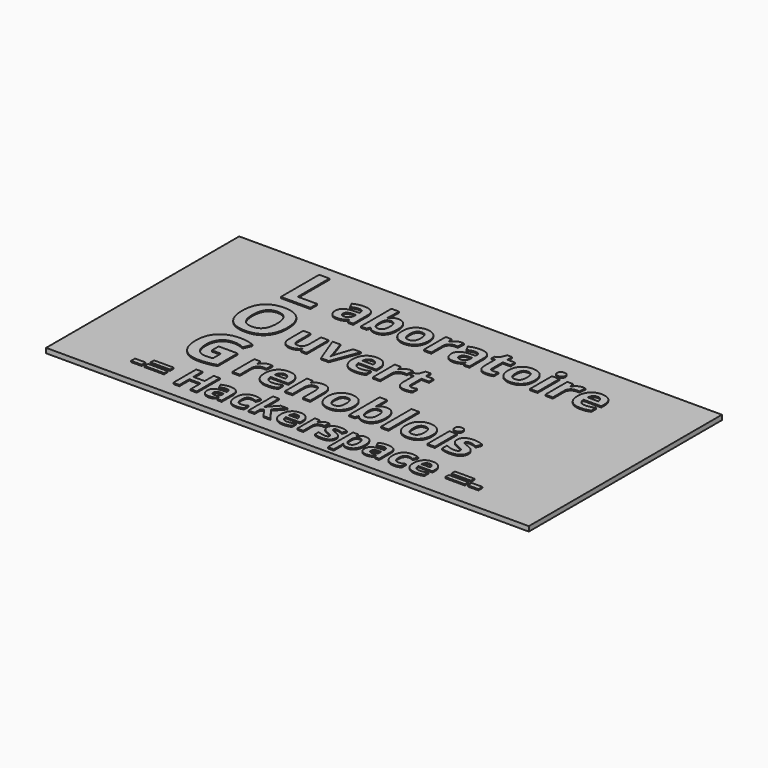
from build123d import *

# Parameters (mm, degrees)
F0_W           = 2000
F0_H           = 1000
F0_W_2         = 43.6979166667
F0_H_2         = 20.3385416667
F0_W_3         = 80.8072916667
F0_H_3         = 17.8385416667
F0_H_4         = 17.8125
F0_W_4         = 31.0221354167
F0_H_5         = 158.30078125
F0_H_6         = 113.7369791667
F0_TEXT_SIZE   = 277.7777777778
F0_TEXT_SIZE_2 = 208.3333333333
F0_TEXT_SIZE_3 = 166.6666666667
F1_DEPTH       = 20
F2_DEPTH       = 5


# Not quite as in the source:
# - Text() gives the source's letters only with a copy of the font that has no kerning and outlines rounded to 1/6400 em; it was checked with that copy


with BuildPart() as f1:
    # F0 (on Top) → F1 (new body)
    with BuildSketch(Plane.XY):
        with Locations((1000, 500)):
            Rectangle(F0_W, F0_H)
        with Locations((299.5572916667, 103.5529597493)):
            Rectangle(F0_W_2, F0_H_2, mode=Mode.SUBTRACT)
        with Locations((373.9192708333, 101.8081680827)):
            Rectangle(F0_W_3, F0_H_3, mode=Mode.SUBTRACT)
        with Locations((373.9192708333, 133.305563916)):
            Rectangle(F0_W_3, F0_H_4, mode=Mode.SUBTRACT)
        Polygon((577.265625, 177.8628555827), (577.265625, 58.8784805827), (552.109375, 58.8784805827), (552.109375, 110.2326472493), (505, 110.2326472493), (505, 58.8784805827), (479.765625, 58.8784805827), (479.765625, 177.8628555827), (505, 177.8628555827), (505, 131.2222305827), (552.109375, 131.2222305827), (552.109375, 177.8628555827), align=None, mode=Mode.SUBTRACT)
        with BuildLine():
            Line((680.4427083333, 58.8784805827), (663.125, 58.8784805827))
            Line((663.125, 58.8784805827), (658.3072916667, 71.2482722493))
            Line((658.3072916667, 71.2482722493), (657.65625, 71.2482722493))
            add(Edge.make_bspline(
                [(657.65625, 71.2482722493), (651.40625, 63.3576472493), (644.765625, 60.297751416)],
                knots=[0, 0, 0, 1, 1, 1], degree=2))
            add(Edge.make_bspline(
                [(644.765625, 60.297751416), (638.125, 57.2378555827), (627.4739583333, 57.2378555827)],
                knots=[0, 0, 0, 1, 1, 1], degree=2))
            add(Edge.make_bspline(
                [(627.4739583333, 57.2378555827), (614.375, 57.2378555827), (606.8489583333, 64.7378555827)],
                knots=[0, 0, 0, 1, 1, 1], degree=2))
            add(Edge.make_bspline(
                [(606.8489583333, 64.7378555827), (599.3229166667, 72.2378555827), (599.3229166667, 86.0659805827)],
                knots=[0, 0, 0, 1, 1, 1], degree=2))
            add(Edge.make_bspline(
                [(599.3229166667, 86.0659805827), (599.3229166667, 100.5451472493), (609.453125, 107.4201472493)],
                knots=[0, 0, 0, 1, 1, 1], degree=2))
            add(Edge.make_bspline(
                [(609.453125, 107.4201472493), (619.5833333333, 114.2951472493), (640, 115.024313916)],
                knots=[0, 0, 0, 1, 1, 1], degree=2))
            Line((640, 115.024313916), (655.8072916667, 115.5191055827))
            Line((655.8072916667, 115.5191055827), (655.8072916667, 119.5034805827))
            add(Edge.make_bspline(
                [(655.8072916667, 119.5034805827), (655.8072916667, 133.3316055827), (641.640625, 133.3316055827)],
                knots=[0, 0, 0, 1, 1, 1], degree=2))
            add(Edge.make_bspline(
                [(641.640625, 133.3316055827), (630.7291666667, 133.3316055827), (615.9895833333, 126.743063916)],
                knots=[0, 0, 0, 1, 1, 1], degree=2))
            Line((615.9895833333, 126.743063916), (607.7864583333, 143.5138972493))
            add(Edge.make_bspline(
                [(607.7864583333, 143.5138972493), (623.4895833333, 151.743063916), (642.6041666667, 151.743063916)],
                knots=[0, 0, 0, 1, 1, 1], degree=2))
            add(Edge.make_bspline(
                [(642.6041666667, 151.743063916), (660.9114583333, 151.743063916), (670.6770833333, 143.7612930827)],
                knots=[0, 0, 0, 1, 1, 1], degree=2))
            add(Edge.make_bspline(
                [(670.6770833333, 143.7612930827), (680.4427083333, 135.7795222493), (680.4427083333, 119.5034805827)],
                knots=[0, 0, 0, 1, 1, 1], degree=2))
            Line((680.4427083333, 119.5034805827), (680.4427083333, 58.8784805827))
        make_face(mode=Mode.SUBTRACT)
        with BuildLine():
            add(Edge.make_bspline(
                [(758.4635416667, 58.7092097493), (752.3177083333, 57.2378555827), (742.96875, 57.2378555827)],
                knots=[0, 0, 0, 1, 1, 1], degree=2))
            add(Edge.make_bspline(
                [(742.96875, 57.2378555827), (700.4947916667, 57.2378555827), (700.4947916667, 103.8784805827)],
                knots=[0, 0, 0, 1, 1, 1], degree=2))
            add(Edge.make_bspline(
                [(700.4947916667, 103.8784805827), (700.4947916667, 127.0816055827), (712.0442708333, 139.321188916)],
                knots=[0, 0, 0, 1, 1, 1], degree=2))
            add(Edge.make_bspline(
                [(712.0442708333, 139.321188916), (723.59375, 151.5607722493), (745.15625, 151.5607722493)],
                knots=[0, 0, 0, 1, 1, 1], degree=2))
            add(Edge.make_bspline(
                [(745.15625, 151.5607722493), (760.9375, 151.5607722493), (773.4895833333, 145.3888972493)],
                knots=[0, 0, 0, 1, 1, 1], degree=2))
            Line((773.4895833333, 145.3888972493), (766.1458333333, 126.1701472493))
            add(Edge.make_bspline(
                [(766.1458333333, 126.1701472493), (760.2864583333, 128.539938916), (755.2473958333, 130.0503555827)],
                knots=[0, 0, 0, 1, 1, 1], degree=2))
            add(Edge.make_bspline(
                [(755.2473958333, 130.0503555827), (750.2083333333, 131.5607722493), (745.15625, 131.5607722493)],
                knots=[0, 0, 0, 1, 1, 1], degree=2))
            add(Edge.make_bspline(
                [(745.15625, 131.5607722493), (725.78125, 131.5607722493), (725.78125, 104.0347305827)],
                knots=[0, 0, 0, 1, 1, 1], degree=2))
            add(Edge.make_bspline(
                [(725.78125, 104.0347305827), (725.78125, 77.3420222493), (745.15625, 77.3420222493)],
                knots=[0, 0, 0, 1, 1, 1], degree=2))
            add(Edge.make_bspline(
                [(745.15625, 77.3420222493), (752.3177083333, 77.3420222493), (758.4244791667, 79.2560847493)],
                knots=[0, 0, 0, 1, 1, 1], degree=2))
            add(Edge.make_bspline(
                [(758.4244791667, 79.2560847493), (764.53125, 81.1701472493), (770.625, 85.258688916)],
                knots=[0, 0, 0, 1, 1, 1], degree=2))
            Line((770.625, 85.258688916), (770.625, 64.008688916))
            add(Edge.make_bspline(
                [(770.625, 64.008688916), (764.609375, 60.180563916), (758.4635416667, 58.7092097493)],
                knots=[0, 0, 0, 1, 1, 1], degree=2))
        make_face(mode=Mode.SUBTRACT)
        Polygon((815.234375, 108.3576472493), (815.5729166667, 108.3576472493), (826.3802083333, 122.1857722493), (851.8489583333, 149.868063916), (879.84375, 149.868063916), (843.7239583333, 110.3888972493), (882.0572916667, 58.8784805827), (853.4114583333, 58.8784805827), (827.2135416667, 95.7534805827), (816.5364583333, 87.211813916), (816.5364583333, 58.8784805827), (791.71875, 58.8784805827), (791.71875, 185.5191055827), (816.5364583333, 185.5191055827), (816.5364583333, 129.0347305827), align=None, mode=Mode.SUBTRACT)
        with BuildLine():
            add(Edge.make_bspline(
                [(954.3229166667, 58.8263972493), (946.9270833333, 57.2378555827), (936.25, 57.2378555827)],
                knots=[0, 0, 0, 1, 1, 1], degree=2))
            add(Edge.make_bspline(
                [(936.25, 57.2378555827), (914.296875, 57.2378555827), (901.9270833333, 69.3732722493)],
                knots=[0, 0, 0, 1, 1, 1], degree=2))
            add(Edge.make_bspline(
                [(901.9270833333, 69.3732722493), (889.5572916667, 81.508688916), (889.5572916667, 103.7222305827)],
                knots=[0, 0, 0, 1, 1, 1], degree=2))
            add(Edge.make_bspline(
                [(889.5572916667, 103.7222305827), (889.5572916667, 126.586813916), (900.9895833333, 139.0737930827)],
                knots=[0, 0, 0, 1, 1, 1], degree=2))
            add(Edge.make_bspline(
                [(900.9895833333, 139.0737930827), (912.421875, 151.5607722493), (932.6041666667, 151.5607722493)],
                knots=[0, 0, 0, 1, 1, 1], degree=2))
            add(Edge.make_bspline(
                [(932.6041666667, 151.5607722493), (951.875, 151.5607722493), (962.6171875, 140.5842097493)],
                knots=[0, 0, 0, 1, 1, 1], degree=2))
            add(Edge.make_bspline(
                [(962.6171875, 140.5842097493), (973.359375, 129.6076472493), (973.359375, 110.2326472493)],
                knots=[0, 0, 0, 1, 1, 1], degree=2))
            Line((973.359375, 110.2326472493), (973.359375, 98.1753555827))
            Line((973.359375, 98.1753555827), (914.6875, 98.1753555827))
            add(Edge.make_bspline(
                [(914.6875, 98.1753555827), (915.1041666667, 87.602438916), (920.9635416667, 81.664938916)],
                knots=[0, 0, 0, 1, 1, 1], degree=2))
            add(Edge.make_bspline(
                [(920.9635416667, 81.664938916), (926.8229166667, 75.727438916), (937.3958333333, 75.727438916)],
                knots=[0, 0, 0, 1, 1, 1], degree=2))
            add(Edge.make_bspline(
                [(937.3958333333, 75.727438916), (945.625, 75.727438916), (952.9427083333, 77.4331680827)],
                knots=[0, 0, 0, 1, 1, 1], degree=2))
            add(Edge.make_bspline(
                [(952.9427083333, 77.4331680827), (960.2604166667, 79.1388972493), (968.2291666667, 82.8888972493)],
                knots=[0, 0, 0, 1, 1, 1], degree=2))
            Line((968.2291666667, 82.8888972493), (968.2291666667, 63.6701472493))
            add(Edge.make_bspline(
                [(968.2291666667, 63.6701472493), (961.71875, 60.414938916), (954.3229166667, 58.8263972493)],
                knots=[0, 0, 0, 1, 1, 1], degree=2))
        make_face(mode=Mode.SUBTRACT)
        with BuildLine():
            Line((435.5729166667, 314.1024472765), (435.5729166667, 349.1284889431))
            Line((435.5729166667, 349.1284889431), (514.2621527778, 349.1284889431))
            Line((514.2621527778, 349.1284889431), (514.2621527778, 246.3073083876))
            add(Edge.make_bspline(
                [(514.2621527778, 246.3073083876), (495.1215277778, 240.0573083876), (478.2378472222, 237.5399472765)],
                knots=[0, 0, 0, 1, 1, 1], degree=2))
            add(Edge.make_bspline(
                [(478.2378472222, 237.5399472765), (461.3541666667, 235.0225861654), (443.7326388889, 235.0225861654)],
                knots=[0, 0, 0, 1, 1, 1], degree=2))
            add(Edge.make_bspline(
                [(443.7326388889, 235.0225861654), (398.8541666667, 235.0225861654), (375.1779513889, 261.4114750543)],
                knots=[0, 0, 0, 1, 1, 1], degree=2))
            add(Edge.make_bspline(
                [(375.1779513889, 261.4114750543), (351.5017361111, 287.8003639431), (351.5017361111, 337.1927250543)],
                knots=[0, 0, 0, 1, 1, 1], degree=2))
            add(Edge.make_bspline(
                [(351.5017361111, 337.1927250543), (351.5017361111, 385.1961972765), (378.9756944444, 412.040815332)],
                knots=[0, 0, 0, 1, 1, 1], degree=2))
            add(Edge.make_bspline(
                [(378.9756944444, 412.040815332), (406.4496527778, 438.8854333876), (455.1041666667, 438.8854333876)],
                knots=[0, 0, 0, 1, 1, 1], degree=2))
            add(Edge.make_bspline(
                [(455.1041666667, 438.8854333876), (485.6597222222, 438.8854333876), (514.0017361111, 426.689252832)],
                knots=[0, 0, 0, 1, 1, 1], degree=2))
            Line((514.0017361111, 426.689252832), (500.0260416667, 393.0521000543))
            add(Edge.make_bspline(
                [(500.0260416667, 393.0521000543), (478.3246527778, 403.9027944987), (454.84375, 403.9027944987)],
                knots=[0, 0, 0, 1, 1, 1], degree=2))
            add(Edge.make_bspline(
                [(454.84375, 403.9027944987), (427.5868055556, 403.9027944987), (411.1805555556, 385.5868222765)],
                knots=[0, 0, 0, 1, 1, 1], degree=2))
            add(Edge.make_bspline(
                [(411.1805555556, 385.5868222765), (394.7743055556, 367.2708500543), (394.7743055556, 336.3680722765)],
                knots=[0, 0, 0, 1, 1, 1], degree=2))
            add(Edge.make_bspline(
                [(394.7743055556, 336.3680722765), (394.7743055556, 304.0764056098), (407.9904513889, 287.0625167209)],
                knots=[0, 0, 0, 1, 1, 1], degree=2))
            add(Edge.make_bspline(
                [(407.9904513889, 287.0625167209), (421.2065972222, 270.048627832), (446.4236111111, 270.048627832)],
                knots=[0, 0, 0, 1, 1, 1], degree=2))
            add(Edge.make_bspline(
                [(446.4236111111, 270.048627832), (459.6180555556, 270.048627832), (473.1597222222, 272.7396000543)],
                knots=[0, 0, 0, 1, 1, 1], degree=2))
            Line((473.1597222222, 272.7396000543), (473.1597222222, 314.1024472765))
            Line((473.1597222222, 314.1024472765), (435.5729166667, 314.1024472765))
        make_face(mode=Mode.SUBTRACT)
        with BuildLine():
            add(Edge.make_bspline(
                [(625.4676649306, 347.7667267904), (634.4683159722, 353.6098257487), (645.0477430556, 353.6098257487)],
                knots=[0, 0, 0, 1, 1, 1], degree=2))
            add(Edge.make_bspline(
                [(645.0477430556, 353.6098257487), (651.3628472222, 353.6098257487), (655.5295138889, 352.6983674154)],
                knots=[0, 0, 0, 1, 1, 1], degree=2))
            Line((655.5295138889, 352.6983674154), (653.1857638889, 323.6293569987))
            add(Edge.make_bspline(
                [(653.1857638889, 323.6293569987), (649.4097222222, 324.638471582), (644.0386284722, 324.638471582)],
                knots=[0, 0, 0, 1, 1, 1], degree=2))
            add(Edge.make_bspline(
                [(644.0386284722, 324.638471582), (629.1948784722, 324.638471582), (620.8940972222, 317.0050080404)],
                knots=[0, 0, 0, 1, 1, 1], degree=2))
            add(Edge.make_bspline(
                [(620.8940972222, 317.0050080404), (612.5933159722, 309.3715444987), (612.5933159722, 295.634565332)],
                knots=[0, 0, 0, 1, 1, 1], degree=2))
            Line((612.5933159722, 295.634565332), (612.5933159722, 237.7569611654))
            Line((612.5933159722, 237.7569611654), (581.5711805556, 237.7569611654))
            Line((581.5711805556, 237.7569611654), (581.5711805556, 351.493940332))
            Line((581.5711805556, 351.493940332), (605.0737847222, 351.493940332))
            Line((605.0737847222, 351.493940332), (609.6636284722, 332.353315332))
            Line((609.6636284722, 332.353315332), (611.1610243056, 332.353315332))
            add(Edge.make_bspline(
                [(611.1610243056, 332.353315332), (616.4670138889, 341.923627832), (625.4676649306, 347.7667267904)],
                knots=[0, 0, 0, 1, 1, 1], degree=2))
        make_face(mode=Mode.SUBTRACT)
        with BuildLine():
            add(Edge.make_bspline(
                [(750.2235243056, 237.6918569987), (740.9787326389, 235.7061799154), (727.6323784722, 235.7061799154)],
                knots=[0, 0, 0, 1, 1, 1], degree=2))
            add(Edge.make_bspline(
                [(727.6323784722, 235.7061799154), (700.1909722222, 235.7061799154), (684.7287326389, 250.8754507487)],
                knots=[0, 0, 0, 1, 1, 1], degree=2))
            add(Edge.make_bspline(
                [(684.7287326389, 250.8754507487), (669.2664930556, 266.044721582), (669.2664930556, 293.8116486654)],
                knots=[0, 0, 0, 1, 1, 1], degree=2))
            add(Edge.make_bspline(
                [(669.2664930556, 293.8116486654), (669.2664930556, 322.392377832), (683.5568576389, 338.0011017904)],
                knots=[0, 0, 0, 1, 1, 1], degree=2))
            add(Edge.make_bspline(
                [(683.5568576389, 338.0011017904), (697.8472222222, 353.6098257487), (723.0750868056, 353.6098257487)],
                knots=[0, 0, 0, 1, 1, 1], degree=2))
            add(Edge.make_bspline(
                [(723.0750868056, 353.6098257487), (747.1636284722, 353.6098257487), (760.5913628472, 339.8891226237)],
                knots=[0, 0, 0, 1, 1, 1], degree=2))
            add(Edge.make_bspline(
                [(760.5913628472, 339.8891226237), (774.0190972222, 326.1684194987), (774.0190972222, 301.9496694987)],
                knots=[0, 0, 0, 1, 1, 1], degree=2))
            Line((774.0190972222, 301.9496694987), (774.0190972222, 286.8780549154))
            Line((774.0190972222, 286.8780549154), (700.6792534722, 286.8780549154))
            add(Edge.make_bspline(
                [(700.6792534722, 286.8780549154), (701.2000868056, 273.661909082), (708.5243055556, 266.240034082)],
                knots=[0, 0, 0, 1, 1, 1], degree=2))
            add(Edge.make_bspline(
                [(708.5243055556, 266.240034082), (715.8485243056, 258.818159082), (729.0646701389, 258.818159082)],
                knots=[0, 0, 0, 1, 1, 1], degree=2))
            add(Edge.make_bspline(
                [(729.0646701389, 258.818159082), (739.3511284722, 258.818159082), (748.4982638889, 260.9503205404)],
                knots=[0, 0, 0, 1, 1, 1], degree=2))
            add(Edge.make_bspline(
                [(748.4982638889, 260.9503205404), (757.6453993056, 263.0824819987), (767.6063368056, 267.7699819987)],
                knots=[0, 0, 0, 1, 1, 1], degree=2))
            Line((767.6063368056, 267.7699819987), (767.6063368056, 243.7465444987))
            add(Edge.make_bspline(
                [(767.6063368056, 243.7465444987), (759.4683159722, 239.677534082), (750.2235243056, 237.6918569987)],
                knots=[0, 0, 0, 1, 1, 1], degree=2))
        make_face(mode=Mode.SUBTRACT)
        with BuildLine():
            Line((904.2274305556, 311.9106069987), (904.2274305556, 237.7569611654))
            Line((904.2274305556, 237.7569611654), (873.2052951389, 237.7569611654))
            Line((873.2052951389, 237.7569611654), (873.2052951389, 304.1957632487))
            add(Edge.make_bspline(
                [(873.2052951389, 304.1957632487), (873.2052951389, 316.5004507487), (868.8270399306, 322.6527944987)],
                knots=[0, 0, 0, 1, 1, 1], degree=2))
            add(Edge.make_bspline(
                [(868.8270399306, 322.6527944987), (864.4487847222, 328.8051382487), (854.8784722222, 328.8051382487)],
                knots=[0, 0, 0, 1, 1, 1], degree=2))
            add(Edge.make_bspline(
                [(854.8784722222, 328.8051382487), (841.8576388889, 328.8051382487), (836.0633680556, 320.1137319987)],
                knots=[0, 0, 0, 1, 1, 1], degree=2))
            add(Edge.make_bspline(
                [(836.0633680556, 320.1137319987), (830.2690972222, 311.4223257487), (830.2690972222, 291.2725861654)],
                knots=[0, 0, 0, 1, 1, 1], degree=2))
            Line((830.2690972222, 291.2725861654), (830.2690972222, 237.7569611654))
            Line((830.2690972222, 237.7569611654), (799.2469618056, 237.7569611654))
            Line((799.2469618056, 237.7569611654), (799.2469618056, 351.493940332))
            Line((799.2469618056, 351.493940332), (822.9448784722, 351.493940332))
            Line((822.9448784722, 351.493940332), (827.1115451389, 336.943159082))
            Line((827.1115451389, 336.943159082), (828.8368055556, 336.943159082))
            add(Edge.make_bspline(
                [(828.8368055556, 336.943159082), (834.0451388889, 345.1788361654), (843.1434461806, 349.394330957)],
                knots=[0, 0, 0, 1, 1, 1], degree=2))
            add(Edge.make_bspline(
                [(843.1434461806, 349.394330957), (852.2417534722, 353.6098257487), (863.8302951389, 353.6098257487)],
                knots=[0, 0, 0, 1, 1, 1], degree=2))
            add(Edge.make_bspline(
                [(863.8302951389, 353.6098257487), (883.6870659722, 353.6098257487), (893.9572482639, 342.8839142904)],
                knots=[0, 0, 0, 1, 1, 1], degree=2))
            add(Edge.make_bspline(
                [(893.9572482639, 342.8839142904), (904.2274305556, 332.158002832), (904.2274305556, 311.9106069987)],
                knots=[0, 0, 0, 1, 1, 1], degree=2))
        make_face(mode=Mode.SUBTRACT)
        with BuildLine():
            add(Edge.make_bspline(
                [(1032.8081597222, 326.054487207), (1039.5138888889, 312.724409082), (1039.5138888889, 294.8207632487)],
                knots=[0, 0, 0, 1, 1, 1], degree=2))
            add(Edge.make_bspline(
                [(1039.5138888889, 294.8207632487), (1039.5138888889, 267.0538361654), (1024.8654513889, 251.3800080404)],
                knots=[0, 0, 0, 1, 1, 1], degree=2))
            add(Edge.make_bspline(
                [(1024.8654513889, 251.3800080404), (1010.2170138889, 235.7061799154), (984.0776909722, 235.7061799154)],
                knots=[0, 0, 0, 1, 1, 1], degree=2))
            add(Edge.make_bspline(
                [(984.0776909722, 235.7061799154), (967.7039930556, 235.7061799154), (955.1877170139, 242.8839142904)],
                knots=[0, 0, 0, 1, 1, 1], degree=2))
            add(Edge.make_bspline(
                [(955.1877170139, 242.8839142904), (942.6714409722, 250.0616486654), (935.9657118056, 263.4893830404)],
                knots=[0, 0, 0, 1, 1, 1], degree=2))
            add(Edge.make_bspline(
                [(935.9657118056, 263.4893830404), (929.2599826389, 276.9171174154), (929.2599826389, 294.8207632487)],
                knots=[0, 0, 0, 1, 1, 1], degree=2))
            add(Edge.make_bspline(
                [(929.2599826389, 294.8207632487), (929.2599826389, 322.685346582), (943.7944878472, 338.1475861654)],
                knots=[0, 0, 0, 1, 1, 1], degree=2))
            add(Edge.make_bspline(
                [(943.7944878472, 338.1475861654), (958.3289930556, 353.6098257487), (984.6961805556, 353.6098257487)],
                knots=[0, 0, 0, 1, 1, 1], degree=2))
            add(Edge.make_bspline(
                [(984.6961805556, 353.6098257487), (1001.0698784722, 353.6098257487), (1013.5861545139, 346.4971955404)],
                knots=[0, 0, 0, 1, 1, 1], degree=2))
            add(Edge.make_bspline(
                [(1013.5861545139, 346.4971955404), (1026.1024305556, 339.384565332), (1032.8081597222, 326.054487207)],
                knots=[0, 0, 0, 1, 1, 1], degree=2))
        make_face(mode=Mode.SUBTRACT)
        with BuildLine():
            add(Edge.make_bspline(
                [(1028.6588541667, 146.8862930827), (1035.859375, 151.5607722493), (1044.3229166667, 151.5607722493)],
                knots=[0, 0, 0, 1, 1, 1], degree=2))
            add(Edge.make_bspline(
                [(1044.3229166667, 151.5607722493), (1049.375, 151.5607722493), (1052.7083333333, 150.8316055827)],
                knots=[0, 0, 0, 1, 1, 1], degree=2))
            Line((1052.7083333333, 150.8316055827), (1050.8333333333, 127.5763972493))
            add(Edge.make_bspline(
                [(1050.8333333333, 127.5763972493), (1047.8125, 128.383688916), (1043.515625, 128.383688916)],
                knots=[0, 0, 0, 1, 1, 1], degree=2))
            add(Edge.make_bspline(
                [(1043.515625, 128.383688916), (1031.640625, 128.383688916), (1025, 122.2769180827)],
                knots=[0, 0, 0, 1, 1, 1], degree=2))
            add(Edge.make_bspline(
                [(1025, 122.2769180827), (1018.359375, 116.1701472493), (1018.359375, 105.180563916)],
                knots=[0, 0, 0, 1, 1, 1], degree=2))
            Line((1018.359375, 105.180563916), (1018.359375, 58.8784805827))
            Line((1018.359375, 58.8784805827), (993.5416666667, 58.8784805827))
            Line((993.5416666667, 58.8784805827), (993.5416666667, 149.868063916))
            Line((993.5416666667, 149.868063916), (1012.34375, 149.868063916))
            Line((1012.34375, 149.868063916), (1016.015625, 134.555563916))
            Line((1016.015625, 134.555563916), (1017.2135416667, 134.555563916))
            add(Edge.make_bspline(
                [(1017.2135416667, 134.555563916), (1021.4583333333, 142.211813916), (1028.6588541667, 146.8862930827)],
                knots=[0, 0, 0, 1, 1, 1], degree=2))
        make_face(mode=Mode.SUBTRACT)
        with BuildLine():
            add(Edge.make_bspline(
                [(1130.3385416667, 97.5373347493), (1132.7083333333, 92.6545222493), (1132.7083333333, 85.9097305827)],
                knots=[0, 0, 0, 1, 1, 1], degree=2))
            add(Edge.make_bspline(
                [(1132.7083333333, 85.9097305827), (1132.7083333333, 71.899313916), (1122.9817708333, 64.5685847493)],
                knots=[0, 0, 0, 1, 1, 1], degree=2))
            add(Edge.make_bspline(
                [(1122.9817708333, 64.5685847493), (1113.2552083333, 57.2378555827), (1093.8802083333, 57.2378555827)],
                knots=[0, 0, 0, 1, 1, 1], degree=2))
            add(Edge.make_bspline(
                [(1093.8802083333, 57.2378555827), (1083.9583333333, 57.2378555827), (1076.953125, 58.5920222493)],
                knots=[0, 0, 0, 1, 1, 1], degree=2))
            add(Edge.make_bspline(
                [(1076.953125, 58.5920222493), (1069.9479166667, 59.946188916), (1063.8541666667, 62.5503555827)],
                knots=[0, 0, 0, 1, 1, 1], degree=2))
            Line((1063.8541666667, 62.5503555827), (1063.8541666667, 83.0451472493))
            add(Edge.make_bspline(
                [(1063.8541666667, 83.0451472493), (1070.7552083333, 79.789938916), (1079.4270833333, 77.5894180827)],
                knots=[0, 0, 0, 1, 1, 1], degree=2))
            add(Edge.make_bspline(
                [(1079.4270833333, 77.5894180827), (1088.0989583333, 75.3888972493), (1094.6875, 75.3888972493)],
                knots=[0, 0, 0, 1, 1, 1], degree=2))
            add(Edge.make_bspline(
                [(1094.6875, 75.3888972493), (1108.203125, 75.3888972493), (1108.203125, 83.2013972493)],
                knots=[0, 0, 0, 1, 1, 1], degree=2))
            add(Edge.make_bspline(
                [(1108.203125, 83.2013972493), (1108.203125, 86.1441055827), (1106.40625, 87.9800430827)],
                knots=[0, 0, 0, 1, 1, 1], degree=2))
            add(Edge.make_bspline(
                [(1106.40625, 87.9800430827), (1104.609375, 89.8159805827), (1100.2213541667, 92.133688916)],
                knots=[0, 0, 0, 1, 1, 1], degree=2))
            add(Edge.make_bspline(
                [(1100.2213541667, 92.133688916), (1095.8333333333, 94.4513972493), (1088.515625, 97.524313916)],
                knots=[0, 0, 0, 1, 1, 1], degree=2))
            add(Edge.make_bspline(
                [(1088.515625, 97.524313916), (1078.0208333333, 101.9253555827), (1073.0859375, 105.6753555827)],
                knots=[0, 0, 0, 1, 1, 1], degree=2))
            add(Edge.make_bspline(
                [(1073.0859375, 105.6753555827), (1068.1510416667, 109.4253555827), (1065.9244791667, 114.2691055827)],
                knots=[0, 0, 0, 1, 1, 1], degree=2))
            add(Edge.make_bspline(
                [(1065.9244791667, 114.2691055827), (1063.6979166667, 119.1128555827), (1063.6979166667, 126.1701472493)],
                knots=[0, 0, 0, 1, 1, 1], degree=2))
            add(Edge.make_bspline(
                [(1063.6979166667, 126.1701472493), (1063.6979166667, 138.305563916), (1073.0859375, 144.9331680827)],
                knots=[0, 0, 0, 1, 1, 1], degree=2))
            add(Edge.make_bspline(
                [(1073.0859375, 144.9331680827), (1082.4739583333, 151.5607722493), (1099.7395833333, 151.5607722493)],
                knots=[0, 0, 0, 1, 1, 1], degree=2))
            add(Edge.make_bspline(
                [(1099.7395833333, 151.5607722493), (1116.171875, 151.5607722493), (1131.71875, 144.399313916)],
                knots=[0, 0, 0, 1, 1, 1], degree=2))
            Line((1131.71875, 144.399313916), (1124.2447916667, 126.508688916))
            add(Edge.make_bspline(
                [(1124.2447916667, 126.508688916), (1117.3958333333, 129.4253555827), (1111.4583333333, 131.3003555827)],
                knots=[0, 0, 0, 1, 1, 1], degree=2))
            add(Edge.make_bspline(
                [(1111.4583333333, 131.3003555827), (1105.5208333333, 133.1753555827), (1099.3229166667, 133.1753555827)],
                knots=[0, 0, 0, 1, 1, 1], degree=2))
            add(Edge.make_bspline(
                [(1099.3229166667, 133.1753555827), (1088.3333333333, 133.1753555827), (1088.3333333333, 127.2378555827)],
                knots=[0, 0, 0, 1, 1, 1], degree=2))
            add(Edge.make_bspline(
                [(1088.3333333333, 127.2378555827), (1088.3333333333, 123.9045222493), (1091.875, 121.4566055827)],
                knots=[0, 0, 0, 1, 1, 1], degree=2))
            add(Edge.make_bspline(
                [(1091.875, 121.4566055827), (1095.4166666667, 119.008688916), (1107.3958333333, 114.2170222493)],
                knots=[0, 0, 0, 1, 1, 1], degree=2))
            add(Edge.make_bspline(
                [(1107.3958333333, 114.2170222493), (1118.046875, 109.8941055827), (1123.0078125, 106.157126416)],
                knots=[0, 0, 0, 1, 1, 1], degree=2))
            add(Edge.make_bspline(
                [(1123.0078125, 106.157126416), (1127.96875, 102.4201472493), (1130.3385416667, 97.5373347493)],
                knots=[0, 0, 0, 1, 1, 1], degree=2))
        make_face(mode=Mode.SUBTRACT)
        with BuildLine():
            add(Edge.make_bspline(
                [(1220.5729166667, 62.8628555827), (1212.6822916667, 57.2378555827), (1202.03125, 57.2378555827)],
                knots=[0, 0, 0, 1, 1, 1], degree=2))
            add(Edge.make_bspline(
                [(1202.03125, 57.2378555827), (1185.9895833333, 57.2378555827), (1176.875, 68.8784805827)],
                knots=[0, 0, 0, 1, 1, 1], degree=2))
            Line((1176.875, 68.8784805827), (1175.5729166667, 68.8784805827))
            add(Edge.make_bspline(
                [(1175.5729166667, 68.8784805827), (1176.875, 57.4982722493), (1176.875, 55.7013972493)],
                knots=[0, 0, 0, 1, 1, 1], degree=2))
            Line((1176.875, 55.7013972493), (1176.875, 18.8263972493))
            Line((1176.875, 18.8263972493), (1152.0572916667, 18.8263972493))
            Line((1152.0572916667, 18.8263972493), (1152.0572916667, 149.868063916))
            Line((1152.0572916667, 149.868063916), (1172.2395833333, 149.868063916))
            Line((1172.2395833333, 149.868063916), (1175.7291666667, 138.071188916))
            Line((1175.7291666667, 138.071188916), (1176.875, 138.071188916))
            add(Edge.make_bspline(
                [(1176.875, 138.071188916), (1185.5989583333, 151.5607722493), (1202.6822916667, 151.5607722493)],
                knots=[0, 0, 0, 1, 1, 1], degree=2))
            add(Edge.make_bspline(
                [(1202.6822916667, 151.5607722493), (1218.8020833333, 151.5607722493), (1227.9166666667, 139.1128555827)],
                knots=[0, 0, 0, 1, 1, 1], degree=2))
            add(Edge.make_bspline(
                [(1227.9166666667, 139.1128555827), (1237.03125, 126.664938916), (1237.03125, 104.5295222493)],
                knots=[0, 0, 0, 1, 1, 1], degree=2))
            add(Edge.make_bspline(
                [(1237.03125, 104.5295222493), (1237.03125, 89.9722305827), (1232.7473958333, 79.2300430827)],
                knots=[0, 0, 0, 1, 1, 1], degree=2))
            add(Edge.make_bspline(
                [(1232.7473958333, 79.2300430827), (1228.4635416667, 68.4878555827), (1220.5729166667, 62.8628555827)],
                knots=[0, 0, 0, 1, 1, 1], degree=2))
        make_face(mode=Mode.SUBTRACT)
        with BuildLine():
            Line((1332.6302083333, 58.8784805827), (1315.3125, 58.8784805827))
            Line((1315.3125, 58.8784805827), (1310.4947916667, 71.2482722493))
            Line((1310.4947916667, 71.2482722493), (1309.84375, 71.2482722493))
            add(Edge.make_bspline(
                [(1309.84375, 71.2482722493), (1303.59375, 63.3576472493), (1296.953125, 60.297751416)],
                knots=[0, 0, 0, 1, 1, 1], degree=2))
            add(Edge.make_bspline(
                [(1296.953125, 60.297751416), (1290.3125, 57.2378555827), (1279.6614583333, 57.2378555827)],
                knots=[0, 0, 0, 1, 1, 1], degree=2))
            add(Edge.make_bspline(
                [(1279.6614583333, 57.2378555827), (1266.5625, 57.2378555827), (1259.0364583333, 64.7378555827)],
                knots=[0, 0, 0, 1, 1, 1], degree=2))
            add(Edge.make_bspline(
                [(1259.0364583333, 64.7378555827), (1251.5104166667, 72.2378555827), (1251.5104166667, 86.0659805827)],
                knots=[0, 0, 0, 1, 1, 1], degree=2))
            add(Edge.make_bspline(
                [(1251.5104166667, 86.0659805827), (1251.5104166667, 100.5451472493), (1261.640625, 107.4201472493)],
                knots=[0, 0, 0, 1, 1, 1], degree=2))
            add(Edge.make_bspline(
                [(1261.640625, 107.4201472493), (1271.7708333333, 114.2951472493), (1292.1875, 115.024313916)],
                knots=[0, 0, 0, 1, 1, 1], degree=2))
            Line((1292.1875, 115.024313916), (1307.9947916667, 115.5191055827))
            Line((1307.9947916667, 115.5191055827), (1307.9947916667, 119.5034805827))
            add(Edge.make_bspline(
                [(1307.9947916667, 119.5034805827), (1307.9947916667, 133.3316055827), (1293.828125, 133.3316055827)],
                knots=[0, 0, 0, 1, 1, 1], degree=2))
            add(Edge.make_bspline(
                [(1293.828125, 133.3316055827), (1282.9166666667, 133.3316055827), (1268.1770833333, 126.743063916)],
                knots=[0, 0, 0, 1, 1, 1], degree=2))
            Line((1268.1770833333, 126.743063916), (1259.9739583333, 143.5138972493))
            add(Edge.make_bspline(
                [(1259.9739583333, 143.5138972493), (1275.6770833333, 151.743063916), (1294.7916666667, 151.743063916)],
                knots=[0, 0, 0, 1, 1, 1], degree=2))
            add(Edge.make_bspline(
                [(1294.7916666667, 151.743063916), (1313.0989583333, 151.743063916), (1322.8645833333, 143.7612930827)],
                knots=[0, 0, 0, 1, 1, 1], degree=2))
            add(Edge.make_bspline(
                [(1322.8645833333, 143.7612930827), (1332.6302083333, 135.7795222493), (1332.6302083333, 119.5034805827)],
                knots=[0, 0, 0, 1, 1, 1], degree=2))
            Line((1332.6302083333, 119.5034805827), (1332.6302083333, 58.8784805827))
        make_face(mode=Mode.SUBTRACT)
        with BuildLine():
            add(Edge.make_bspline(
                [(1410.6510416667, 58.7092097493), (1404.5052083333, 57.2378555827), (1395.15625, 57.2378555827)],
                knots=[0, 0, 0, 1, 1, 1], degree=2))
            add(Edge.make_bspline(
                [(1395.15625, 57.2378555827), (1352.6822916667, 57.2378555827), (1352.6822916667, 103.8784805827)],
                knots=[0, 0, 0, 1, 1, 1], degree=2))
            add(Edge.make_bspline(
                [(1352.6822916667, 103.8784805827), (1352.6822916667, 127.0816055827), (1364.2317708333, 139.321188916)],
                knots=[0, 0, 0, 1, 1, 1], degree=2))
            add(Edge.make_bspline(
                [(1364.2317708333, 139.321188916), (1375.78125, 151.5607722493), (1397.34375, 151.5607722493)],
                knots=[0, 0, 0, 1, 1, 1], degree=2))
            add(Edge.make_bspline(
                [(1397.34375, 151.5607722493), (1413.125, 151.5607722493), (1425.6770833333, 145.3888972493)],
                knots=[0, 0, 0, 1, 1, 1], degree=2))
            Line((1425.6770833333, 145.3888972493), (1418.3333333333, 126.1701472493))
            add(Edge.make_bspline(
                [(1418.3333333333, 126.1701472493), (1412.4739583333, 128.539938916), (1407.4348958333, 130.0503555827)],
                knots=[0, 0, 0, 1, 1, 1], degree=2))
            add(Edge.make_bspline(
                [(1407.4348958333, 130.0503555827), (1402.3958333333, 131.5607722493), (1397.34375, 131.5607722493)],
                knots=[0, 0, 0, 1, 1, 1], degree=2))
            add(Edge.make_bspline(
                [(1397.34375, 131.5607722493), (1377.96875, 131.5607722493), (1377.96875, 104.0347305827)],
                knots=[0, 0, 0, 1, 1, 1], degree=2))
            add(Edge.make_bspline(
                [(1377.96875, 104.0347305827), (1377.96875, 77.3420222493), (1397.34375, 77.3420222493)],
                knots=[0, 0, 0, 1, 1, 1], degree=2))
            add(Edge.make_bspline(
                [(1397.34375, 77.3420222493), (1404.5052083333, 77.3420222493), (1410.6119791667, 79.2560847493)],
                knots=[0, 0, 0, 1, 1, 1], degree=2))
            add(Edge.make_bspline(
                [(1410.6119791667, 79.2560847493), (1416.71875, 81.1701472493), (1422.8125, 85.258688916)],
                knots=[0, 0, 0, 1, 1, 1], degree=2))
            Line((1422.8125, 85.258688916), (1422.8125, 64.008688916))
            add(Edge.make_bspline(
                [(1422.8125, 64.008688916), (1416.796875, 60.180563916), (1410.6510416667, 58.7092097493)],
                knots=[0, 0, 0, 1, 1, 1], degree=2))
        make_face(mode=Mode.SUBTRACT)
        with BuildLine():
            add(Edge.make_bspline(
                [(1503.1510416667, 58.8263972493), (1495.7552083333, 57.2378555827), (1485.078125, 57.2378555827)],
                knots=[0, 0, 0, 1, 1, 1], degree=2))
            add(Edge.make_bspline(
                [(1485.078125, 57.2378555827), (1463.125, 57.2378555827), (1450.7552083333, 69.3732722493)],
                knots=[0, 0, 0, 1, 1, 1], degree=2))
            add(Edge.make_bspline(
                [(1450.7552083333, 69.3732722493), (1438.3854166667, 81.508688916), (1438.3854166667, 103.7222305827)],
                knots=[0, 0, 0, 1, 1, 1], degree=2))
            add(Edge.make_bspline(
                [(1438.3854166667, 103.7222305827), (1438.3854166667, 126.586813916), (1449.8177083333, 139.0737930827)],
                knots=[0, 0, 0, 1, 1, 1], degree=2))
            add(Edge.make_bspline(
                [(1449.8177083333, 139.0737930827), (1461.25, 151.5607722493), (1481.4322916667, 151.5607722493)],
                knots=[0, 0, 0, 1, 1, 1], degree=2))
            add(Edge.make_bspline(
                [(1481.4322916667, 151.5607722493), (1500.703125, 151.5607722493), (1511.4453125, 140.5842097493)],
                knots=[0, 0, 0, 1, 1, 1], degree=2))
            add(Edge.make_bspline(
                [(1511.4453125, 140.5842097493), (1522.1875, 129.6076472493), (1522.1875, 110.2326472493)],
                knots=[0, 0, 0, 1, 1, 1], degree=2))
            Line((1522.1875, 110.2326472493), (1522.1875, 98.1753555827))
            Line((1522.1875, 98.1753555827), (1463.515625, 98.1753555827))
            add(Edge.make_bspline(
                [(1463.515625, 98.1753555827), (1463.9322916667, 87.602438916), (1469.7916666667, 81.664938916)],
                knots=[0, 0, 0, 1, 1, 1], degree=2))
            add(Edge.make_bspline(
                [(1469.7916666667, 81.664938916), (1475.6510416667, 75.727438916), (1486.2239583333, 75.727438916)],
                knots=[0, 0, 0, 1, 1, 1], degree=2))
            add(Edge.make_bspline(
                [(1486.2239583333, 75.727438916), (1494.453125, 75.727438916), (1501.7708333333, 77.4331680827)],
                knots=[0, 0, 0, 1, 1, 1], degree=2))
            add(Edge.make_bspline(
                [(1501.7708333333, 77.4331680827), (1509.0885416667, 79.1388972493), (1517.0572916667, 82.8888972493)],
                knots=[0, 0, 0, 1, 1, 1], degree=2))
            Line((1517.0572916667, 82.8888972493), (1517.0572916667, 63.6701472493))
            add(Edge.make_bspline(
                [(1517.0572916667, 63.6701472493), (1510.546875, 60.414938916), (1503.1510416667, 58.8263972493)],
                knots=[0, 0, 0, 1, 1, 1], degree=2))
        make_face(mode=Mode.SUBTRACT)
        with Locations((1620.2213541667, 101.8081680827)):
            Rectangle(F0_W_3, F0_H_3, mode=Mode.SUBTRACT)
        with Locations((1694.609375, 103.5529597493)):
            Rectangle(F0_W_2, F0_H_2, mode=Mode.SUBTRACT)
        with Locations((1620.2213541667, 133.305563916)):
            Rectangle(F0_W_3, F0_H_4, mode=Mode.SUBTRACT)
        with BuildLine():
            add(Edge.make_bspline(
                [(1096.1870659722, 336.747846582), (1107.0920138889, 353.6098257487), (1128.4461805556, 353.6098257487)],
                knots=[0, 0, 0, 1, 1, 1], degree=2))
            add(Edge.make_bspline(
                [(1128.4461805556, 353.6098257487), (1148.5959201389, 353.6098257487), (1159.9891493056, 337.9034455404)],
                knots=[0, 0, 0, 1, 1, 1], degree=2))
            add(Edge.make_bspline(
                [(1159.9891493056, 337.9034455404), (1171.3823784722, 322.197065332), (1171.3823784722, 294.8207632487)],
                knots=[0, 0, 0, 1, 1, 1], degree=2))
            add(Edge.make_bspline(
                [(1171.3823784722, 294.8207632487), (1171.3823784722, 266.6632111654), (1159.6310763889, 251.1846955404)],
                knots=[0, 0, 0, 1, 1, 1], degree=2))
            add(Edge.make_bspline(
                [(1159.6310763889, 251.1846955404), (1147.8797743056, 235.7061799154), (1127.6323784722, 235.7061799154)],
                knots=[0, 0, 0, 1, 1, 1], degree=2))
            add(Edge.make_bspline(
                [(1127.6323784722, 235.7061799154), (1107.5802951389, 235.7061799154), (1096.1870659722, 250.2569611654)],
                knots=[0, 0, 0, 1, 1, 1], degree=2))
            Line((1096.1870659722, 250.2569611654), (1094.0711805556, 250.2569611654))
            Line((1094.0711805556, 250.2569611654), (1088.8628472222, 237.7569611654))
            Line((1088.8628472222, 237.7569611654), (1065.1649305556, 237.7569611654))
            Line((1065.1649305556, 237.7569611654), (1065.1649305556, 396.0577424154))
            Line((1065.1649305556, 396.0577424154), (1096.1870659722, 396.0577424154))
            Line((1096.1870659722, 396.0577424154), (1096.1870659722, 359.208784082))
            add(Edge.make_bspline(
                [(1096.1870659722, 359.208784082), (1096.1870659722, 352.2100861654), (1094.9826388889, 336.747846582)],
                knots=[0, 0, 0, 1, 1, 1], degree=2))
            Line((1094.9826388889, 336.747846582), (1096.1870659722, 336.747846582))
        make_face(mode=Mode.SUBTRACT)
        with Locations((1212.5119357639, 316.9073517904)):
            Rectangle(F0_W_4, F0_H_5, mode=Mode.SUBTRACT)
        with BuildLine():
            add(Edge.make_bspline(
                [(1357.2222222222, 326.054487207), (1363.9279513889, 312.724409082), (1363.9279513889, 294.8207632487)],
                knots=[0, 0, 0, 1, 1, 1], degree=2))
            add(Edge.make_bspline(
                [(1363.9279513889, 294.8207632487), (1363.9279513889, 267.0538361654), (1349.2795138889, 251.3800080404)],
                knots=[0, 0, 0, 1, 1, 1], degree=2))
            add(Edge.make_bspline(
                [(1349.2795138889, 251.3800080404), (1334.6310763889, 235.7061799154), (1308.4917534722, 235.7061799154)],
                knots=[0, 0, 0, 1, 1, 1], degree=2))
            add(Edge.make_bspline(
                [(1308.4917534722, 235.7061799154), (1292.1180555556, 235.7061799154), (1279.6017795139, 242.8839142904)],
                knots=[0, 0, 0, 1, 1, 1], degree=2))
            add(Edge.make_bspline(
                [(1279.6017795139, 242.8839142904), (1267.0855034722, 250.0616486654), (1260.3797743056, 263.4893830404)],
                knots=[0, 0, 0, 1, 1, 1], degree=2))
            add(Edge.make_bspline(
                [(1260.3797743056, 263.4893830404), (1253.6740451389, 276.9171174154), (1253.6740451389, 294.8207632487)],
                knots=[0, 0, 0, 1, 1, 1], degree=2))
            add(Edge.make_bspline(
                [(1253.6740451389, 294.8207632487), (1253.6740451389, 322.685346582), (1268.2085503472, 338.1475861654)],
                knots=[0, 0, 0, 1, 1, 1], degree=2))
            add(Edge.make_bspline(
                [(1268.2085503472, 338.1475861654), (1282.7430555556, 353.6098257487), (1309.1102430556, 353.6098257487)],
                knots=[0, 0, 0, 1, 1, 1], degree=2))
            add(Edge.make_bspline(
                [(1309.1102430556, 353.6098257487), (1325.4839409722, 353.6098257487), (1338.0002170139, 346.4971955404)],
                knots=[0, 0, 0, 1, 1, 1], degree=2))
            add(Edge.make_bspline(
                [(1338.0002170139, 346.4971955404), (1350.5164930556, 339.384565332), (1357.2222222222, 326.054487207)],
                knots=[0, 0, 0, 1, 1, 1], degree=2))
        make_face(mode=Mode.SUBTRACT)
        with Locations((1405.0900607639, 294.6254507487)):
            Rectangle(F0_W_4, F0_H_6, mode=Mode.SUBTRACT)
        with BuildLine():
            add(Edge.make_bspline(
                [(1529.5529513889, 286.0805288737), (1532.5151909722, 279.9770132487), (1532.5151909722, 271.5460236654)],
                knots=[0, 0, 0, 1, 1, 1], degree=2))
            add(Edge.make_bspline(
                [(1532.5151909722, 271.5460236654), (1532.5151909722, 254.033002832), (1520.3569878472, 244.8695913737)],
                knots=[0, 0, 0, 1, 1, 1], degree=2))
            add(Edge.make_bspline(
                [(1520.3569878472, 244.8695913737), (1508.1987847222, 235.7061799154), (1483.9800347222, 235.7061799154)],
                knots=[0, 0, 0, 1, 1, 1], degree=2))
            add(Edge.make_bspline(
                [(1483.9800347222, 235.7061799154), (1471.5776909722, 235.7061799154), (1462.8211805556, 237.3988882487)],
                knots=[0, 0, 0, 1, 1, 1], degree=2))
            add(Edge.make_bspline(
                [(1462.8211805556, 237.3988882487), (1454.0646701389, 239.091596582), (1446.4474826389, 242.3468049154)],
                knots=[0, 0, 0, 1, 1, 1], degree=2))
            Line((1446.4474826389, 242.3468049154), (1446.4474826389, 267.9652944987))
            add(Edge.make_bspline(
                [(1446.4474826389, 267.9652944987), (1455.0737847222, 263.896284082), (1465.9136284722, 261.1456330404)],
                knots=[0, 0, 0, 1, 1, 1], degree=2))
            add(Edge.make_bspline(
                [(1465.9136284722, 261.1456330404), (1476.7534722222, 258.3949819987), (1484.9891493056, 258.3949819987)],
                knots=[0, 0, 0, 1, 1, 1], degree=2))
            add(Edge.make_bspline(
                [(1484.9891493056, 258.3949819987), (1501.8836805556, 258.3949819987), (1501.8836805556, 268.1606069987)],
                knots=[0, 0, 0, 1, 1, 1], degree=2))
            add(Edge.make_bspline(
                [(1501.8836805556, 268.1606069987), (1501.8836805556, 271.8389924154), (1499.6375868056, 274.1339142904)],
                knots=[0, 0, 0, 1, 1, 1], degree=2))
            add(Edge.make_bspline(
                [(1499.6375868056, 274.1339142904), (1497.3914930556, 276.4288361654), (1491.9064670139, 279.325971582)],
                knots=[0, 0, 0, 1, 1, 1], degree=2))
            add(Edge.make_bspline(
                [(1491.9064670139, 279.325971582), (1486.4214409722, 282.2231069987), (1477.2743055556, 286.064252832)],
                knots=[0, 0, 0, 1, 1, 1], degree=2))
            add(Edge.make_bspline(
                [(1477.2743055556, 286.064252832), (1464.1558159722, 291.5655549154), (1457.9871961806, 296.2530549154)],
                knots=[0, 0, 0, 1, 1, 1], degree=2))
            add(Edge.make_bspline(
                [(1457.9871961806, 296.2530549154), (1451.8185763889, 300.9405549154), (1449.0353732639, 306.9952424154)],
                knots=[0, 0, 0, 1, 1, 1], degree=2))
            add(Edge.make_bspline(
                [(1449.0353732639, 306.9952424154), (1446.2521701389, 313.0499299154), (1446.2521701389, 321.8715444987)],
                knots=[0, 0, 0, 1, 1, 1], degree=2))
            add(Edge.make_bspline(
                [(1446.2521701389, 321.8715444987), (1446.2521701389, 337.040815332), (1457.9871961806, 345.3253205404)],
                knots=[0, 0, 0, 1, 1, 1], degree=2))
            add(Edge.make_bspline(
                [(1457.9871961806, 345.3253205404), (1469.7222222222, 353.6098257487), (1491.3042534722, 353.6098257487)],
                knots=[0, 0, 0, 1, 1, 1], degree=2))
            add(Edge.make_bspline(
                [(1491.3042534722, 353.6098257487), (1511.8446180556, 353.6098257487), (1531.2782118056, 344.658002832)],
                knots=[0, 0, 0, 1, 1, 1], degree=2))
            Line((1531.2782118056, 344.658002832), (1521.9357638889, 322.294721582))
            add(Edge.make_bspline(
                [(1521.9357638889, 322.294721582), (1513.3745659722, 325.9405549154), (1505.9526909722, 328.2843049154)],
                knots=[0, 0, 0, 1, 1, 1], degree=2))
            add(Edge.make_bspline(
                [(1505.9526909722, 328.2843049154), (1498.5308159722, 330.6280549154), (1490.7834201389, 330.6280549154)],
                knots=[0, 0, 0, 1, 1, 1], degree=2))
            add(Edge.make_bspline(
                [(1490.7834201389, 330.6280549154), (1477.0464409722, 330.6280549154), (1477.0464409722, 323.2061799154)],
                knots=[0, 0, 0, 1, 1, 1], degree=2))
            add(Edge.make_bspline(
                [(1477.0464409722, 323.2061799154), (1477.0464409722, 319.0395132487), (1481.4735243056, 315.9796174154)],
                knots=[0, 0, 0, 1, 1, 1], degree=2))
            add(Edge.make_bspline(
                [(1481.4735243056, 315.9796174154), (1485.9006076389, 312.919721582), (1500.8745659722, 306.9301382487)],
                knots=[0, 0, 0, 1, 1, 1], degree=2))
            add(Edge.make_bspline(
                [(1500.8745659722, 306.9301382487), (1514.1883680556, 301.5264924154), (1520.3895399306, 296.855268457)],
                knots=[0, 0, 0, 1, 1, 1], degree=2))
            add(Edge.make_bspline(
                [(1520.3895399306, 296.855268457), (1526.5907118056, 292.1840444987), (1529.5529513889, 286.0805288737)],
                knots=[0, 0, 0, 1, 1, 1], degree=2))
        make_face(mode=Mode.SUBTRACT)
        with BuildLine():
            add(Edge.make_bspline(
                [(1405.1388888889, 365.6215444987), (1388.2443576389, 365.6215444987), (1388.2443576389, 380.888471582)],
                knots=[0, 0, 0, 1, 1, 1], degree=2))
            add(Edge.make_bspline(
                [(1388.2443576389, 380.888471582), (1388.2443576389, 396.0577424154), (1405.1388888889, 396.0577424154)],
                knots=[0, 0, 0, 1, 1, 1], degree=2))
            add(Edge.make_bspline(
                [(1405.1388888889, 396.0577424154), (1422.0334201389, 396.0577424154), (1422.0334201389, 380.888471582)],
                knots=[0, 0, 0, 1, 1, 1], degree=2))
            add(Edge.make_bspline(
                [(1422.0334201389, 380.888471582), (1422.0334201389, 373.661909082), (1417.8179253472, 369.6417267904)],
                knots=[0, 0, 0, 1, 1, 1], degree=2))
            add(Edge.make_bspline(
                [(1417.8179253472, 369.6417267904), (1413.6024305556, 365.6215444987), (1405.1388888889, 365.6215444987)],
                knots=[0, 0, 0, 1, 1, 1], degree=2))
        make_face(mode=Mode.SUBTRACT)
        with BuildLine():
            add(Edge.make_bspline(
                [(503.0642361111, 666.9464810547), (527.2829861111, 640.6226963325), (527.2829861111, 591.2737379991)],
                knots=[0, 0, 0, 1, 1, 1], degree=2))
            add(Edge.make_bspline(
                [(527.2829861111, 591.2737379991), (527.2829861111, 542.0115852214), (502.8689236111, 515.5575921658)],
                knots=[0, 0, 0, 1, 1, 1], degree=2))
            add(Edge.make_bspline(
                [(502.8689236111, 515.5575921658), (478.4548611111, 489.1035991102), (432.8819444444, 489.1035991102)],
                knots=[0, 0, 0, 1, 1, 1], degree=2))
            add(Edge.make_bspline(
                [(432.8819444444, 489.1035991102), (387.3090277778, 489.1035991102), (362.8949652778, 515.5575921658)],
                knots=[0, 0, 0, 1, 1, 1], degree=2))
            add(Edge.make_bspline(
                [(362.8949652778, 515.5575921658), (338.4809027778, 542.0115852214), (338.4809027778, 591.5341546658)],
                knots=[0, 0, 0, 1, 1, 1], degree=2))
            add(Edge.make_bspline(
                [(338.4809027778, 591.5341546658), (338.4809027778, 641.0567241102), (362.9600694444, 667.1634949436)],
                knots=[0, 0, 0, 1, 1, 1], degree=2))
            add(Edge.make_bspline(
                [(362.9600694444, 667.1634949436), (387.4392361111, 693.2702657769), (433.1423611111, 693.2702657769)],
                knots=[0, 0, 0, 1, 1, 1], degree=2))
            add(Edge.make_bspline(
                [(433.1423611111, 693.2702657769), (478.8454861111, 693.2702657769), (503.0642361111, 666.9464810547)],
                knots=[0, 0, 0, 1, 1, 1], degree=2))
        make_face(mode=Mode.SUBTRACT)
        with BuildLine():
            Line((685.9331597222, 491.8379741102), (662.1375868056, 491.8379741102))
            Line((662.1375868056, 491.8379741102), (657.9709201389, 506.3887553602))
            Line((657.9709201389, 506.3887553602), (656.3433159722, 506.3887553602))
            add(Edge.make_bspline(
                [(656.3433159722, 506.3887553602), (651.3628472222, 498.4460470269), (642.1994357639, 494.1166199436)],
                knots=[0, 0, 0, 1, 1, 1], degree=2))
            add(Edge.make_bspline(
                [(642.1994357639, 494.1166199436), (633.0360243056, 489.7871928602), (621.3498263889, 489.7871928602)],
                knots=[0, 0, 0, 1, 1, 1], degree=2))
            add(Edge.make_bspline(
                [(621.3498263889, 489.7871928602), (601.2977430556, 489.7871928602), (591.1252170139, 500.5293803602)],
                knots=[0, 0, 0, 1, 1, 1], degree=2))
            add(Edge.make_bspline(
                [(591.1252170139, 500.5293803602), (580.9526909722, 511.2715678602), (580.9526909722, 531.4213074436)],
                knots=[0, 0, 0, 1, 1, 1], degree=2))
            Line((580.9526909722, 531.4213074436), (580.9526909722, 605.5749532769))
            Line((580.9526909722, 605.5749532769), (611.9748263889, 605.5749532769))
            Line((611.9748263889, 605.5749532769), (611.9748263889, 539.1361511936))
            add(Edge.make_bspline(
                [(611.9748263889, 539.1361511936), (611.9748263889, 526.8314636936), (616.3530815972, 520.6791199436)],
                knots=[0, 0, 0, 1, 1, 1], degree=2))
            add(Edge.make_bspline(
                [(616.3530815972, 520.6791199436), (620.7313368056, 514.5267761936), (630.3016493056, 514.5267761936)],
                knots=[0, 0, 0, 1, 1, 1], degree=2))
            add(Edge.make_bspline(
                [(630.3016493056, 514.5267761936), (643.3224826389, 514.5267761936), (649.1167534722, 523.2181824436)],
                knots=[0, 0, 0, 1, 1, 1], degree=2))
            add(Edge.make_bspline(
                [(649.1167534722, 523.2181824436), (654.9110243056, 531.9095886936), (654.9110243056, 552.0593282769)],
                knots=[0, 0, 0, 1, 1, 1], degree=2))
            Line((654.9110243056, 552.0593282769), (654.9110243056, 605.5749532769))
            Line((654.9110243056, 605.5749532769), (685.9331597222, 605.5749532769))
            Line((685.9331597222, 605.5749532769), (685.9331597222, 491.8379741102))
        make_face(mode=Mode.SUBTRACT)
        with BuildLine():
            Line((777.3719618056, 491.8379741102), (745.5360243056, 491.8379741102))
            Line((745.5360243056, 491.8379741102), (702.2092013889, 605.5749532769))
            Line((702.2092013889, 605.5749532769), (734.6636284722, 605.5749532769))
            Line((734.6636284722, 605.5749532769), (756.6362847222, 540.7637553602))
            add(Edge.make_bspline(
                [(756.6362847222, 540.7637553602), (760.2821180556, 528.4590678602), (761.2261284722, 517.4890157769)],
                knots=[0, 0, 0, 1, 1, 1], degree=2))
            Line((761.2261284722, 517.4890157769), (761.8120659722, 517.4890157769))
            add(Edge.make_bspline(
                [(761.8120659722, 517.4890157769), (762.3328993056, 527.2546407769), (766.4019097222, 540.7637553602)],
                knots=[0, 0, 0, 1, 1, 1], degree=2))
            Line((766.4019097222, 540.7637553602), (788.2769097222, 605.5749532769))
            Line((788.2769097222, 605.5749532769), (820.7313368056, 605.5749532769))
            Line((820.7313368056, 605.5749532769), (777.3719618056, 491.8379741102))
        make_face(mode=Mode.SUBTRACT)
        with BuildLine():
            add(Edge.make_bspline(
                [(911.0633680556, 491.7728699436), (901.8185763889, 489.7871928602), (888.4722222222, 489.7871928602)],
                knots=[0, 0, 0, 1, 1, 1], degree=2))
            add(Edge.make_bspline(
                [(888.4722222222, 489.7871928602), (861.0308159722, 489.7871928602), (845.5685763889, 504.9564636936)],
                knots=[0, 0, 0, 1, 1, 1], degree=2))
            add(Edge.make_bspline(
                [(845.5685763889, 504.9564636936), (830.1063368056, 520.1257345269), (830.1063368056, 547.8926616102)],
                knots=[0, 0, 0, 1, 1, 1], degree=2))
            add(Edge.make_bspline(
                [(830.1063368056, 547.8926616102), (830.1063368056, 576.4733907769), (844.3967013889, 592.0821147352)],
                knots=[0, 0, 0, 1, 1, 1], degree=2))
            add(Edge.make_bspline(
                [(844.3967013889, 592.0821147352), (858.6870659722, 607.6908386936), (883.9149305556, 607.6908386936)],
                knots=[0, 0, 0, 1, 1, 1], degree=2))
            add(Edge.make_bspline(
                [(883.9149305556, 607.6908386936), (908.0034722222, 607.6908386936), (921.4312065972, 593.9701355686)],
                knots=[0, 0, 0, 1, 1, 1], degree=2))
            add(Edge.make_bspline(
                [(921.4312065972, 593.9701355686), (934.8589409722, 580.2494324436), (934.8589409722, 556.0306824436)],
                knots=[0, 0, 0, 1, 1, 1], degree=2))
            Line((934.8589409722, 556.0306824436), (934.8589409722, 540.9590678602))
            Line((934.8589409722, 540.9590678602), (861.5190972222, 540.9590678602))
            add(Edge.make_bspline(
                [(861.5190972222, 540.9590678602), (862.0399305556, 527.7429220269), (869.3641493056, 520.3210470269)],
                knots=[0, 0, 0, 1, 1, 1], degree=2))
            add(Edge.make_bspline(
                [(869.3641493056, 520.3210470269), (876.6883680556, 512.8991720269), (889.9045138889, 512.8991720269)],
                knots=[0, 0, 0, 1, 1, 1], degree=2))
            add(Edge.make_bspline(
                [(889.9045138889, 512.8991720269), (900.1909722222, 512.8991720269), (909.3381076389, 515.0313334852)],
                knots=[0, 0, 0, 1, 1, 1], degree=2))
            add(Edge.make_bspline(
                [(909.3381076389, 515.0313334852), (918.4852430556, 517.1634949436), (928.4461805556, 521.8509949436)],
                knots=[0, 0, 0, 1, 1, 1], degree=2))
            Line((928.4461805556, 521.8509949436), (928.4461805556, 497.8275574436))
            add(Edge.make_bspline(
                [(928.4461805556, 497.8275574436), (920.3081597222, 493.7585470269), (911.0633680556, 491.7728699436)],
                knots=[0, 0, 0, 1, 1, 1], degree=2))
        make_face(mode=Mode.SUBTRACT)
        with BuildLine():
            add(Edge.make_bspline(
                [(1003.9832899306, 601.8477397352), (1012.9839409722, 607.6908386936), (1023.5633680556, 607.6908386936)],
                knots=[0, 0, 0, 1, 1, 1], degree=2))
            add(Edge.make_bspline(
                [(1023.5633680556, 607.6908386936), (1029.8784722222, 607.6908386936), (1034.0451388889, 606.7793803602)],
                knots=[0, 0, 0, 1, 1, 1], degree=2))
            Line((1034.0451388889, 606.7793803602), (1031.7013888889, 577.7103699436))
            add(Edge.make_bspline(
                [(1031.7013888889, 577.7103699436), (1027.9253472222, 578.7194845269), (1022.5542534722, 578.7194845269)],
                knots=[0, 0, 0, 1, 1, 1], degree=2))
            add(Edge.make_bspline(
                [(1022.5542534722, 578.7194845269), (1007.7105034722, 578.7194845269), (999.4097222222, 571.0860209852)],
                knots=[0, 0, 0, 1, 1, 1], degree=2))
            add(Edge.make_bspline(
                [(999.4097222222, 571.0860209852), (991.1089409722, 563.4525574436), (991.1089409722, 549.7155782769)],
                knots=[0, 0, 0, 1, 1, 1], degree=2))
            Line((991.1089409722, 549.7155782769), (991.1089409722, 491.8379741102))
            Line((991.1089409722, 491.8379741102), (960.0868055556, 491.8379741102))
            Line((960.0868055556, 491.8379741102), (960.0868055556, 605.5749532769))
            Line((960.0868055556, 605.5749532769), (983.5894097222, 605.5749532769))
            Line((983.5894097222, 605.5749532769), (988.1792534722, 586.4343282769))
            Line((988.1792534722, 586.4343282769), (989.6766493056, 586.4343282769))
            add(Edge.make_bspline(
                [(989.6766493056, 586.4343282769), (994.9826388889, 596.0046407769), (1003.9832899306, 601.8477397352)],
                knots=[0, 0, 0, 1, 1, 1], degree=2))
        make_face(mode=Mode.SUBTRACT)
        Polygon((498.5286458333, 745.9189870551), (376.0460069444, 745.9189870551), (376.0460069444, 944.2262787218), (418.1032986111, 944.2262787218), (418.1032986111, 780.6412092773), (498.5286458333, 780.6412092773), align=None, mode=Mode.SUBTRACT)
        with BuildLine():
            Line((675.4513888889, 745.9189870551), (653.8042534722, 745.9189870551))
            Line((653.8042534722, 745.9189870551), (647.7821180556, 761.3812266385))
            Line((647.7821180556, 761.3812266385), (646.9683159722, 761.3812266385))
            add(Edge.make_bspline(
                [(646.9683159722, 761.3812266385), (639.1558159722, 751.5179453885), (630.8550347222, 747.6930755968)],
                knots=[0, 0, 0, 1, 1, 1], degree=2))
            add(Edge.make_bspline(
                [(630.8550347222, 747.6930755968), (622.5542534722, 743.8682058051), (609.2404513889, 743.8682058051)],
                knots=[0, 0, 0, 1, 1, 1], degree=2))
            add(Edge.make_bspline(
                [(609.2404513889, 743.8682058051), (592.8667534722, 743.8682058051), (583.4592013889, 753.2432058051)],
                knots=[0, 0, 0, 1, 1, 1], degree=2))
            add(Edge.make_bspline(
                [(583.4592013889, 753.2432058051), (574.0516493056, 762.6182058051), (574.0516493056, 779.9033620551)],
                knots=[0, 0, 0, 1, 1, 1], degree=2))
            add(Edge.make_bspline(
                [(574.0516493056, 779.9033620551), (574.0516493056, 798.0023203885), (586.7144097222, 806.5960703885)],
                knots=[0, 0, 0, 1, 1, 1], degree=2))
            add(Edge.make_bspline(
                [(586.7144097222, 806.5960703885), (599.3771701389, 815.1898203885), (624.8980034722, 816.1012787218)],
                knots=[0, 0, 0, 1, 1, 1], degree=2))
            Line((624.8980034722, 816.1012787218), (644.6571180556, 816.7197683051))
            Line((644.6571180556, 816.7197683051), (644.6571180556, 821.7002370551))
            add(Edge.make_bspline(
                [(644.6571180556, 821.7002370551), (644.6571180556, 838.9853933051), (626.9487847222, 838.9853933051)],
                knots=[0, 0, 0, 1, 1, 1], degree=2))
            add(Edge.make_bspline(
                [(626.9487847222, 838.9853933051), (613.3094618056, 838.9853933051), (594.8849826389, 830.7497162218)],
                knots=[0, 0, 0, 1, 1, 1], degree=2))
            Line((594.8849826389, 830.7497162218), (584.6310763889, 851.7132578885))
            add(Edge.make_bspline(
                [(584.6310763889, 851.7132578885), (604.2599826389, 861.9997162218), (628.1532118056, 861.9997162218)],
                knots=[0, 0, 0, 1, 1, 1], degree=2))
            add(Edge.make_bspline(
                [(628.1532118056, 861.9997162218), (651.0373263889, 861.9997162218), (663.2443576389, 852.0225026801)],
                knots=[0, 0, 0, 1, 1, 1], degree=2))
            add(Edge.make_bspline(
                [(663.2443576389, 852.0225026801), (675.4513888889, 842.0452891385), (675.4513888889, 821.7002370551)],
                knots=[0, 0, 0, 1, 1, 1], degree=2))
            Line((675.4513888889, 821.7002370551), (675.4513888889, 745.9189870551))
        make_face(mode=Mode.SUBTRACT)
        with BuildLine():
            add(Edge.make_bspline(
                [(935.9006076389, 834.2165130968), (942.6063368056, 820.8864349718), (942.6063368056, 802.9827891385)],
                knots=[0, 0, 0, 1, 1, 1], degree=2))
            add(Edge.make_bspline(
                [(942.6063368056, 802.9827891385), (942.6063368056, 775.2158620551), (927.9578993056, 759.5420339301)],
                knots=[0, 0, 0, 1, 1, 1], degree=2))
            add(Edge.make_bspline(
                [(927.9578993056, 759.5420339301), (913.3094618056, 743.8682058051), (887.1701388889, 743.8682058051)],
                knots=[0, 0, 0, 1, 1, 1], degree=2))
            add(Edge.make_bspline(
                [(887.1701388889, 743.8682058051), (870.7964409722, 743.8682058051), (858.2801649306, 751.0459401801)],
                knots=[0, 0, 0, 1, 1, 1], degree=2))
            add(Edge.make_bspline(
                [(858.2801649306, 751.0459401801), (845.7638888889, 758.2236745551), (839.0581597222, 771.6514089301)],
                knots=[0, 0, 0, 1, 1, 1], degree=2))
            add(Edge.make_bspline(
                [(839.0581597222, 771.6514089301), (832.3524305556, 785.0791433051), (832.3524305556, 802.9827891385)],
                knots=[0, 0, 0, 1, 1, 1], degree=2))
            add(Edge.make_bspline(
                [(832.3524305556, 802.9827891385), (832.3524305556, 830.8473724718), (846.8869357639, 846.3096120551)],
                knots=[0, 0, 0, 1, 1, 1], degree=2))
            add(Edge.make_bspline(
                [(846.8869357639, 846.3096120551), (861.4214409722, 861.7718516385), (887.7886284722, 861.7718516385)],
                knots=[0, 0, 0, 1, 1, 1], degree=2))
            add(Edge.make_bspline(
                [(887.7886284722, 861.7718516385), (904.1623263889, 861.7718516385), (916.6786024306, 854.6592214301)],
                knots=[0, 0, 0, 1, 1, 1], degree=2))
            add(Edge.make_bspline(
                [(916.6786024306, 854.6592214301), (929.1948784722, 847.5465912218), (935.9006076389, 834.2165130968)],
                knots=[0, 0, 0, 1, 1, 1], degree=2))
        make_face(mode=Mode.SUBTRACT)
        with BuildLine():
            add(Edge.make_bspline(
                [(738.4396701389, 844.9098724718), (749.3446180556, 861.7718516385), (770.6987847222, 861.7718516385)],
                knots=[0, 0, 0, 1, 1, 1], degree=2))
            add(Edge.make_bspline(
                [(770.6987847222, 861.7718516385), (790.8485243056, 861.7718516385), (802.2417534722, 846.0654714301)],
                knots=[0, 0, 0, 1, 1, 1], degree=2))
            add(Edge.make_bspline(
                [(802.2417534722, 846.0654714301), (813.6349826389, 830.3590912218), (813.6349826389, 802.9827891385)],
                knots=[0, 0, 0, 1, 1, 1], degree=2))
            add(Edge.make_bspline(
                [(813.6349826389, 802.9827891385), (813.6349826389, 774.8252370551), (801.8836805556, 759.3467214301)],
                knots=[0, 0, 0, 1, 1, 1], degree=2))
            add(Edge.make_bspline(
                [(801.8836805556, 759.3467214301), (790.1323784722, 743.8682058051), (769.8849826389, 743.8682058051)],
                knots=[0, 0, 0, 1, 1, 1], degree=2))
            add(Edge.make_bspline(
                [(769.8849826389, 743.8682058051), (749.8328993056, 743.8682058051), (738.4396701389, 758.4189870551)],
                knots=[0, 0, 0, 1, 1, 1], degree=2))
            Line((738.4396701389, 758.4189870551), (736.3237847222, 758.4189870551))
            Line((736.3237847222, 758.4189870551), (731.1154513889, 745.9189870551))
            Line((731.1154513889, 745.9189870551), (707.4175347222, 745.9189870551))
            Line((707.4175347222, 745.9189870551), (707.4175347222, 904.2197683051))
            Line((707.4175347222, 904.2197683051), (738.4396701389, 904.2197683051))
            Line((738.4396701389, 904.2197683051), (738.4396701389, 867.3708099718))
            add(Edge.make_bspline(
                [(738.4396701389, 867.3708099718), (738.4396701389, 860.3721120551), (737.2352430556, 844.9098724718)],
                knots=[0, 0, 0, 1, 1, 1], degree=2))
            Line((737.2352430556, 844.9098724718), (738.4396701389, 844.9098724718))
        make_face(mode=Mode.SUBTRACT)
        with BuildLine():
            add(Edge.make_bspline(
                [(1092.7690972222, 517.6843282769), (1096.4800347222, 514.5267761936), (1102.5998263889, 514.5267761936)],
                knots=[0, 0, 0, 1, 1, 1], degree=2))
            add(Edge.make_bspline(
                [(1102.5998263889, 514.5267761936), (1110.7378472222, 514.5267761936), (1122.1310763889, 518.0749532769)],
                knots=[0, 0, 0, 1, 1, 1], degree=2))
            Line((1122.1310763889, 518.0749532769), (1122.1310763889, 494.9955261936))
            add(Edge.make_bspline(
                [(1122.1310763889, 494.9955261936), (1110.5425347222, 489.7871928602), (1093.6480034722, 489.7871928602)],
                knots=[0, 0, 0, 1, 1, 1], degree=2))
            add(Edge.make_bspline(
                [(1093.6480034722, 489.7871928602), (1075.0282118056, 489.7871928602), (1066.5321180556, 499.2110209852)],
                knots=[0, 0, 0, 1, 1, 1], degree=2))
            add(Edge.make_bspline(
                [(1066.5321180556, 499.2110209852), (1058.0360243056, 508.6348491102), (1058.0360243056, 527.4499532769)],
                knots=[0, 0, 0, 1, 1, 1], degree=2))
            Line((1058.0360243056, 527.4499532769), (1058.0360243056, 582.2676616102))
            Line((1058.0360243056, 582.2676616102), (1043.1922743056, 582.2676616102))
            Line((1043.1922743056, 582.2676616102), (1043.1922743056, 595.3861511936))
            Line((1043.1922743056, 595.3861511936), (1060.2821180556, 605.7702657769))
            Line((1060.2821180556, 605.7702657769), (1069.2339409722, 629.7937032769))
            Line((1069.2339409722, 629.7937032769), (1089.0581597222, 629.7937032769))
            Line((1089.0581597222, 629.7937032769), (1089.0581597222, 605.5749532769))
            Line((1089.0581597222, 605.5749532769), (1120.8940972222, 605.5749532769))
            Line((1120.8940972222, 605.5749532769), (1120.8940972222, 582.2676616102))
            Line((1120.8940972222, 582.2676616102), (1089.0581597222, 582.2676616102))
            Line((1089.0581597222, 582.2676616102), (1089.0581597222, 527.4499532769))
            add(Edge.make_bspline(
                [(1089.0581597222, 527.4499532769), (1089.0581597222, 520.8418803602), (1092.7690972222, 517.6843282769)],
                knots=[0, 0, 0, 1, 1, 1], degree=2))
        make_face(mode=Mode.SUBTRACT)
        with BuildLine():
            add(Edge.make_bspline(
                [(1012.1538628472, 855.9287526801), (1021.1545138889, 861.7718516385), (1031.7339409722, 861.7718516385)],
                knots=[0, 0, 0, 1, 1, 1], degree=2))
            add(Edge.make_bspline(
                [(1031.7339409722, 861.7718516385), (1038.0490451389, 861.7718516385), (1042.2157118056, 860.8603933051)],
                knots=[0, 0, 0, 1, 1, 1], degree=2))
            Line((1042.2157118056, 860.8603933051), (1039.8719618056, 831.7913828885))
            add(Edge.make_bspline(
                [(1039.8719618056, 831.7913828885), (1036.0959201389, 832.8004974718), (1030.7248263889, 832.8004974718)],
                knots=[0, 0, 0, 1, 1, 1], degree=2))
            add(Edge.make_bspline(
                [(1030.7248263889, 832.8004974718), (1015.8810763889, 832.8004974718), (1007.5802951389, 825.1670339301)],
                knots=[0, 0, 0, 1, 1, 1], degree=2))
            add(Edge.make_bspline(
                [(1007.5802951389, 825.1670339301), (999.2795138889, 817.5335703885), (999.2795138889, 803.7965912218)],
                knots=[0, 0, 0, 1, 1, 1], degree=2))
            Line((999.2795138889, 803.7965912218), (999.2795138889, 745.9189870551))
            Line((999.2795138889, 745.9189870551), (968.2573784722, 745.9189870551))
            Line((968.2573784722, 745.9189870551), (968.2573784722, 859.6559662218))
            Line((968.2573784722, 859.6559662218), (991.7599826389, 859.6559662218))
            Line((991.7599826389, 859.6559662218), (996.3498263889, 840.5153412218))
            Line((996.3498263889, 840.5153412218), (997.8472222222, 840.5153412218))
            add(Edge.make_bspline(
                [(997.8472222222, 840.5153412218), (1003.1532118056, 850.0856537218), (1012.1538628472, 855.9287526801)],
                knots=[0, 0, 0, 1, 1, 1], degree=2))
        make_face(mode=Mode.SUBTRACT)
        with BuildLine():
            Line((1156.7339409722, 745.9189870551), (1135.0868055556, 745.9189870551))
            Line((1135.0868055556, 745.9189870551), (1129.0646701389, 761.3812266385))
            Line((1129.0646701389, 761.3812266385), (1128.2508680556, 761.3812266385))
            add(Edge.make_bspline(
                [(1128.2508680556, 761.3812266385), (1120.4383680556, 751.5179453885), (1112.1375868056, 747.6930755968)],
                knots=[0, 0, 0, 1, 1, 1], degree=2))
            add(Edge.make_bspline(
                [(1112.1375868056, 747.6930755968), (1103.8368055556, 743.8682058051), (1090.5230034722, 743.8682058051)],
                knots=[0, 0, 0, 1, 1, 1], degree=2))
            add(Edge.make_bspline(
                [(1090.5230034722, 743.8682058051), (1074.1493055556, 743.8682058051), (1064.7417534722, 753.2432058051)],
                knots=[0, 0, 0, 1, 1, 1], degree=2))
            add(Edge.make_bspline(
                [(1064.7417534722, 753.2432058051), (1055.3342013889, 762.6182058051), (1055.3342013889, 779.9033620551)],
                knots=[0, 0, 0, 1, 1, 1], degree=2))
            add(Edge.make_bspline(
                [(1055.3342013889, 779.9033620551), (1055.3342013889, 798.0023203885), (1067.9969618056, 806.5960703885)],
                knots=[0, 0, 0, 1, 1, 1], degree=2))
            add(Edge.make_bspline(
                [(1067.9969618056, 806.5960703885), (1080.6597222222, 815.1898203885), (1106.1805555556, 816.1012787218)],
                knots=[0, 0, 0, 1, 1, 1], degree=2))
            Line((1106.1805555556, 816.1012787218), (1125.9396701389, 816.7197683051))
            Line((1125.9396701389, 816.7197683051), (1125.9396701389, 821.7002370551))
            add(Edge.make_bspline(
                [(1125.9396701389, 821.7002370551), (1125.9396701389, 838.9853933051), (1108.2313368056, 838.9853933051)],
                knots=[0, 0, 0, 1, 1, 1], degree=2))
            add(Edge.make_bspline(
                [(1108.2313368056, 838.9853933051), (1094.5920138889, 838.9853933051), (1076.1675347222, 830.7497162218)],
                knots=[0, 0, 0, 1, 1, 1], degree=2))
            Line((1076.1675347222, 830.7497162218), (1065.9136284722, 851.7132578885))
            add(Edge.make_bspline(
                [(1065.9136284722, 851.7132578885), (1085.5425347222, 861.9997162218), (1109.4357638889, 861.9997162218)],
                knots=[0, 0, 0, 1, 1, 1], degree=2))
            add(Edge.make_bspline(
                [(1109.4357638889, 861.9997162218), (1132.3198784722, 861.9997162218), (1144.5269097222, 852.0225026801)],
                knots=[0, 0, 0, 1, 1, 1], degree=2))
            add(Edge.make_bspline(
                [(1144.5269097222, 852.0225026801), (1156.7339409722, 842.0452891385), (1156.7339409722, 821.7002370551)],
                knots=[0, 0, 0, 1, 1, 1], degree=2))
            Line((1156.7339409722, 821.7002370551), (1156.7339409722, 745.9189870551))
        make_face(mode=Mode.SUBTRACT)
        with BuildLine():
            add(Edge.make_bspline(
                [(1226.7860243056, 771.7653412218), (1230.4969618056, 768.6077891385), (1236.6167534722, 768.6077891385)],
                knots=[0, 0, 0, 1, 1, 1], degree=2))
            add(Edge.make_bspline(
                [(1236.6167534722, 768.6077891385), (1244.7547743056, 768.6077891385), (1256.1480034722, 772.1559662218)],
                knots=[0, 0, 0, 1, 1, 1], degree=2))
            Line((1256.1480034722, 772.1559662218), (1256.1480034722, 749.0765391385))
            add(Edge.make_bspline(
                [(1256.1480034722, 749.0765391385), (1244.5594618056, 743.8682058051), (1227.6649305556, 743.8682058051)],
                knots=[0, 0, 0, 1, 1, 1], degree=2))
            add(Edge.make_bspline(
                [(1227.6649305556, 743.8682058051), (1209.0451388889, 743.8682058051), (1200.5490451389, 753.2920339301)],
                knots=[0, 0, 0, 1, 1, 1], degree=2))
            add(Edge.make_bspline(
                [(1200.5490451389, 753.2920339301), (1192.0529513889, 762.7158620551), (1192.0529513889, 781.5309662218)],
                knots=[0, 0, 0, 1, 1, 1], degree=2))
            Line((1192.0529513889, 781.5309662218), (1192.0529513889, 836.3486745551))
            Line((1192.0529513889, 836.3486745551), (1177.2092013889, 836.3486745551))
            Line((1177.2092013889, 836.3486745551), (1177.2092013889, 849.4671641385))
            Line((1177.2092013889, 849.4671641385), (1194.2990451389, 859.8512787218))
            Line((1194.2990451389, 859.8512787218), (1203.2508680556, 883.8747162218))
            Line((1203.2508680556, 883.8747162218), (1223.0750868056, 883.8747162218))
            Line((1223.0750868056, 883.8747162218), (1223.0750868056, 859.6559662218))
            Line((1223.0750868056, 859.6559662218), (1254.9110243056, 859.6559662218))
            Line((1254.9110243056, 859.6559662218), (1254.9110243056, 836.3486745551))
            Line((1254.9110243056, 836.3486745551), (1223.0750868056, 836.3486745551))
            Line((1223.0750868056, 836.3486745551), (1223.0750868056, 781.5309662218))
            add(Edge.make_bspline(
                [(1223.0750868056, 781.5309662218), (1223.0750868056, 774.9228933051), (1226.7860243056, 771.7653412218)],
                knots=[0, 0, 0, 1, 1, 1], degree=2))
        make_face(mode=Mode.SUBTRACT)
        with BuildLine():
            add(Edge.make_bspline(
                [(1375.7769097222, 834.2165130968), (1382.4826388889, 820.8864349718), (1382.4826388889, 802.9827891385)],
                knots=[0, 0, 0, 1, 1, 1], degree=2))
            add(Edge.make_bspline(
                [(1382.4826388889, 802.9827891385), (1382.4826388889, 775.2158620551), (1367.8342013889, 759.5420339301)],
                knots=[0, 0, 0, 1, 1, 1], degree=2))
            add(Edge.make_bspline(
                [(1367.8342013889, 759.5420339301), (1353.1857638889, 743.8682058051), (1327.0464409722, 743.8682058051)],
                knots=[0, 0, 0, 1, 1, 1], degree=2))
            add(Edge.make_bspline(
                [(1327.0464409722, 743.8682058051), (1310.6727430556, 743.8682058051), (1298.1564670139, 751.0459401801)],
                knots=[0, 0, 0, 1, 1, 1], degree=2))
            add(Edge.make_bspline(
                [(1298.1564670139, 751.0459401801), (1285.6401909722, 758.2236745551), (1278.9344618056, 771.6514089301)],
                knots=[0, 0, 0, 1, 1, 1], degree=2))
            add(Edge.make_bspline(
                [(1278.9344618056, 771.6514089301), (1272.2287326389, 785.0791433051), (1272.2287326389, 802.9827891385)],
                knots=[0, 0, 0, 1, 1, 1], degree=2))
            add(Edge.make_bspline(
                [(1272.2287326389, 802.9827891385), (1272.2287326389, 830.8473724718), (1286.7632378472, 846.3096120551)],
                knots=[0, 0, 0, 1, 1, 1], degree=2))
            add(Edge.make_bspline(
                [(1286.7632378472, 846.3096120551), (1301.2977430556, 861.7718516385), (1327.6649305556, 861.7718516385)],
                knots=[0, 0, 0, 1, 1, 1], degree=2))
            add(Edge.make_bspline(
                [(1327.6649305556, 861.7718516385), (1344.0386284722, 861.7718516385), (1356.5549045139, 854.6592214301)],
                knots=[0, 0, 0, 1, 1, 1], degree=2))
            add(Edge.make_bspline(
                [(1356.5549045139, 854.6592214301), (1369.0711805556, 847.5465912218), (1375.7769097222, 834.2165130968)],
                knots=[0, 0, 0, 1, 1, 1], degree=2))
        make_face(mode=Mode.SUBTRACT)
        with Locations((1423.6447482639, 802.7874766385)):
            Rectangle(F0_W_4, F0_H_6, mode=Mode.SUBTRACT)
        with BuildLine():
            add(Edge.make_bspline(
                [(1423.6935763889, 873.7835703885), (1406.7990451389, 873.7835703885), (1406.7990451389, 889.0504974718)],
                knots=[0, 0, 0, 1, 1, 1], degree=2))
            add(Edge.make_bspline(
                [(1406.7990451389, 889.0504974718), (1406.7990451389, 904.2197683051), (1423.6935763889, 904.2197683051)],
                knots=[0, 0, 0, 1, 1, 1], degree=2))
            add(Edge.make_bspline(
                [(1423.6935763889, 904.2197683051), (1440.5881076389, 904.2197683051), (1440.5881076389, 889.0504974718)],
                knots=[0, 0, 0, 1, 1, 1], degree=2))
            add(Edge.make_bspline(
                [(1440.5881076389, 889.0504974718), (1440.5881076389, 881.8239349718), (1436.3726128472, 877.8037526801)],
                knots=[0, 0, 0, 1, 1, 1], degree=2))
            add(Edge.make_bspline(
                [(1436.3726128472, 877.8037526801), (1432.1571180556, 873.7835703885), (1423.6935763889, 873.7835703885)],
                knots=[0, 0, 0, 1, 1, 1], degree=2))
        make_face(mode=Mode.SUBTRACT)
        with BuildLine():
            add(Edge.make_bspline(
                [(1515.6043836806, 855.9287526801), (1524.6050347222, 861.7718516385), (1535.1844618056, 861.7718516385)],
                knots=[0, 0, 0, 1, 1, 1], degree=2))
            add(Edge.make_bspline(
                [(1535.1844618056, 861.7718516385), (1541.4995659722, 861.7718516385), (1545.6662326389, 860.8603933051)],
                knots=[0, 0, 0, 1, 1, 1], degree=2))
            Line((1545.6662326389, 860.8603933051), (1543.3224826389, 831.7913828885))
            add(Edge.make_bspline(
                [(1543.3224826389, 831.7913828885), (1539.5464409722, 832.8004974718), (1534.1753472222, 832.8004974718)],
                knots=[0, 0, 0, 1, 1, 1], degree=2))
            add(Edge.make_bspline(
                [(1534.1753472222, 832.8004974718), (1519.3315972222, 832.8004974718), (1511.0308159722, 825.1670339301)],
                knots=[0, 0, 0, 1, 1, 1], degree=2))
            add(Edge.make_bspline(
                [(1511.0308159722, 825.1670339301), (1502.7300347222, 817.5335703885), (1502.7300347222, 803.7965912218)],
                knots=[0, 0, 0, 1, 1, 1], degree=2))
            Line((1502.7300347222, 803.7965912218), (1502.7300347222, 745.9189870551))
            Line((1502.7300347222, 745.9189870551), (1471.7078993056, 745.9189870551))
            Line((1471.7078993056, 745.9189870551), (1471.7078993056, 859.6559662218))
            Line((1471.7078993056, 859.6559662218), (1495.2105034722, 859.6559662218))
            Line((1495.2105034722, 859.6559662218), (1499.8003472222, 840.5153412218))
            Line((1499.8003472222, 840.5153412218), (1501.2977430556, 840.5153412218))
            add(Edge.make_bspline(
                [(1501.2977430556, 840.5153412218), (1506.6037326389, 850.0856537218), (1515.6043836806, 855.9287526801)],
                knots=[0, 0, 0, 1, 1, 1], degree=2))
        make_face(mode=Mode.SUBTRACT)
        with BuildLine():
            add(Edge.make_bspline(
                [(1640.3602430556, 745.8538828885), (1631.1154513889, 743.8682058051), (1617.7690972222, 743.8682058051)],
                knots=[0, 0, 0, 1, 1, 1], degree=2))
            add(Edge.make_bspline(
                [(1617.7690972222, 743.8682058051), (1590.3276909722, 743.8682058051), (1574.8654513889, 759.0374766385)],
                knots=[0, 0, 0, 1, 1, 1], degree=2))
            add(Edge.make_bspline(
                [(1574.8654513889, 759.0374766385), (1559.4032118056, 774.2067474718), (1559.4032118056, 801.9736745551)],
                knots=[0, 0, 0, 1, 1, 1], degree=2))
            add(Edge.make_bspline(
                [(1559.4032118056, 801.9736745551), (1559.4032118056, 830.5544037218), (1573.6935763889, 846.1631276801)],
                knots=[0, 0, 0, 1, 1, 1], degree=2))
            add(Edge.make_bspline(
                [(1573.6935763889, 846.1631276801), (1587.9839409722, 861.7718516385), (1613.2118055556, 861.7718516385)],
                knots=[0, 0, 0, 1, 1, 1], degree=2))
            add(Edge.make_bspline(
                [(1613.2118055556, 861.7718516385), (1637.3003472222, 861.7718516385), (1650.7280815972, 848.0511485135)],
                knots=[0, 0, 0, 1, 1, 1], degree=2))
            add(Edge.make_bspline(
                [(1650.7280815972, 848.0511485135), (1664.1558159722, 834.3304453885), (1664.1558159722, 810.1116953885)],
                knots=[0, 0, 0, 1, 1, 1], degree=2))
            Line((1664.1558159722, 810.1116953885), (1664.1558159722, 795.0400808051))
            Line((1664.1558159722, 795.0400808051), (1590.8159722222, 795.0400808051))
            add(Edge.make_bspline(
                [(1590.8159722222, 795.0400808051), (1591.3368055556, 781.8239349718), (1598.6610243056, 774.4020599718)],
                knots=[0, 0, 0, 1, 1, 1], degree=2))
            add(Edge.make_bspline(
                [(1598.6610243056, 774.4020599718), (1605.9852430556, 766.9801849718), (1619.2013888889, 766.9801849718)],
                knots=[0, 0, 0, 1, 1, 1], degree=2))
            add(Edge.make_bspline(
                [(1619.2013888889, 766.9801849718), (1629.4878472222, 766.9801849718), (1638.6349826389, 769.1123464301)],
                knots=[0, 0, 0, 1, 1, 1], degree=2))
            add(Edge.make_bspline(
                [(1638.6349826389, 769.1123464301), (1647.7821180556, 771.2445078885), (1657.7430555556, 775.9320078885)],
                knots=[0, 0, 0, 1, 1, 1], degree=2))
            Line((1657.7430555556, 775.9320078885), (1657.7430555556, 751.9085703885))
            add(Edge.make_bspline(
                [(1657.7430555556, 751.9085703885), (1649.6050347222, 747.8395599718), (1640.3602430556, 745.8538828885)],
                knots=[0, 0, 0, 1, 1, 1], degree=2))
        make_face(mode=Mode.SUBTRACT)
        with Locations((322.3350694444, 491.8379741102)):
            Text('O', F0_TEXT_SIZE, font='Open Sans', font_style=FontStyle.BOLD, text_align=(TextAlign.LEFT, TextAlign.BOTTOM))
        with Locations((335.3559027778, 237.7569611654)):
            Text('G', F0_TEXT_SIZE, font='Open Sans', font_style=FontStyle.BOLD, text_align=(TextAlign.LEFT, TextAlign.BOTTOM))
        with BuildLine():
            add(Edge.make_bspline(
                [(395.3168402778, 641.3605435547), (382.578125, 624.4768629991), (382.578125, 591.2737379991)],
                knots=[0, 0, 0, 1, 1, 1], degree=2))
            add(Edge.make_bspline(
                [(382.578125, 591.2737379991), (382.578125, 558.0272102214), (395.1866319444, 541.2086338325)],
                knots=[0, 0, 0, 1, 1, 1], degree=2))
            add(Edge.make_bspline(
                [(395.1866319444, 541.2086338325), (407.7951388889, 524.3900574436), (432.8819444444, 524.3900574436)],
                knots=[0, 0, 0, 1, 1, 1], degree=2))
            add(Edge.make_bspline(
                [(432.8819444444, 524.3900574436), (483.1857638889, 524.3900574436), (483.1857638889, 591.2737379991)],
                knots=[0, 0, 0, 1, 1, 1], degree=2))
            add(Edge.make_bspline(
                [(483.1857638889, 591.2737379991), (483.1857638889, 658.2442241102), (433.1423611111, 658.2442241102)],
                knots=[0, 0, 0, 1, 1, 1], degree=2))
            add(Edge.make_bspline(
                [(433.1423611111, 658.2442241102), (408.0555555556, 658.2442241102), (395.3168402778, 641.3605435547)],
                knots=[0, 0, 0, 1, 1, 1], degree=2))
        make_face()
        with Locations((351.0894097222, 745.9189870551)):
            Text('L', F0_TEXT_SIZE, font='Open Sans', font_style=FontStyle.BOLD, text_align=(TextAlign.LEFT, TextAlign.BOTTOM))
        with Locations((565.2951388889, 491.8379741102)):
            Text('uvert', F0_TEXT_SIZE_2, font='Open Sans', font_style=FontStyle.BOLD, text_align=(TextAlign.LEFT, TextAlign.BOTTOM))
        with BuildLine():
            add(Edge.make_bspline(
                [(869.4618055556, 828.3734141385), (863.9605034722, 819.9749766385), (863.9605034722, 802.9827891385)],
                knots=[0, 0, 0, 1, 1, 1], degree=2))
            add(Edge.make_bspline(
                [(863.9605034722, 802.9827891385), (863.9605034722, 786.0882578885), (869.5106336806, 777.4456797635)],
                knots=[0, 0, 0, 1, 1, 1], degree=2))
            add(Edge.make_bspline(
                [(869.5106336806, 777.4456797635), (875.0607638889, 768.8031016385), (887.5607638889, 768.8031016385)],
                knots=[0, 0, 0, 1, 1, 1], degree=2))
            add(Edge.make_bspline(
                [(887.5607638889, 768.8031016385), (899.9956597222, 768.8031016385), (905.4318576389, 777.3968516385)],
                knots=[0, 0, 0, 1, 1, 1], degree=2))
            add(Edge.make_bspline(
                [(905.4318576389, 777.3968516385), (910.8680555556, 785.9906016385), (910.8680555556, 802.9827891385)],
                knots=[0, 0, 0, 1, 1, 1], degree=2))
            add(Edge.make_bspline(
                [(910.8680555556, 802.9827891385), (910.8680555556, 819.8773203885), (905.3830295139, 828.3245860135)],
                knots=[0, 0, 0, 1, 1, 1], degree=2))
            add(Edge.make_bspline(
                [(905.3830295139, 828.3245860135), (899.8980034722, 836.7718516385), (887.3654513889, 836.7718516385)],
                knots=[0, 0, 0, 1, 1, 1], degree=2))
            add(Edge.make_bspline(
                [(887.3654513889, 836.7718516385), (874.9631076389, 836.7718516385), (869.4618055556, 828.3734141385)],
                knots=[0, 0, 0, 1, 1, 1], degree=2))
        make_face()
        with BuildLine():
            add(Edge.make_bspline(
                [(1309.3381076389, 828.3734141385), (1303.8368055556, 819.9749766385), (1303.8368055556, 802.9827891385)],
                knots=[0, 0, 0, 1, 1, 1], degree=2))
            add(Edge.make_bspline(
                [(1303.8368055556, 802.9827891385), (1303.8368055556, 786.0882578885), (1309.3869357639, 777.4456797635)],
                knots=[0, 0, 0, 1, 1, 1], degree=2))
            add(Edge.make_bspline(
                [(1309.3869357639, 777.4456797635), (1314.9370659722, 768.8031016385), (1327.4370659722, 768.8031016385)],
                knots=[0, 0, 0, 1, 1, 1], degree=2))
            add(Edge.make_bspline(
                [(1327.4370659722, 768.8031016385), (1339.8719618056, 768.8031016385), (1345.3081597222, 777.3968516385)],
                knots=[0, 0, 0, 1, 1, 1], degree=2))
            add(Edge.make_bspline(
                [(1345.3081597222, 777.3968516385), (1350.7443576389, 785.9906016385), (1350.7443576389, 802.9827891385)],
                knots=[0, 0, 0, 1, 1, 1], degree=2))
            add(Edge.make_bspline(
                [(1350.7443576389, 802.9827891385), (1350.7443576389, 819.8773203885), (1345.2593315972, 828.3245860135)],
                knots=[0, 0, 0, 1, 1, 1], degree=2))
            add(Edge.make_bspline(
                [(1345.2593315972, 828.3245860135), (1339.7743055556, 836.7718516385), (1327.2417534722, 836.7718516385)],
                knots=[0, 0, 0, 1, 1, 1], degree=2))
            add(Edge.make_bspline(
                [(1327.2417534722, 836.7718516385), (1314.8394097222, 836.7718516385), (1309.3381076389, 828.3734141385)],
                knots=[0, 0, 0, 1, 1, 1], degree=2))
        make_face()
        with BuildLine():
            add(Edge.make_bspline(
                [(966.3693576389, 320.2113882487), (960.8680555556, 311.8129507487), (960.8680555556, 294.8207632487)],
                knots=[0, 0, 0, 1, 1, 1], degree=2))
            add(Edge.make_bspline(
                [(960.8680555556, 294.8207632487), (960.8680555556, 277.9262319987), (966.4181857639, 269.2836538737)],
                knots=[0, 0, 0, 1, 1, 1], degree=2))
            add(Edge.make_bspline(
                [(966.4181857639, 269.2836538737), (971.9683159722, 260.6410757487), (984.4683159722, 260.6410757487)],
                knots=[0, 0, 0, 1, 1, 1], degree=2))
            add(Edge.make_bspline(
                [(984.4683159722, 260.6410757487), (996.9032118056, 260.6410757487), (1002.3394097222, 269.2348257487)],
                knots=[0, 0, 0, 1, 1, 1], degree=2))
            add(Edge.make_bspline(
                [(1002.3394097222, 269.2348257487), (1007.7756076389, 277.8285757487), (1007.7756076389, 294.8207632487)],
                knots=[0, 0, 0, 1, 1, 1], degree=2))
            add(Edge.make_bspline(
                [(1007.7756076389, 294.8207632487), (1007.7756076389, 311.7152944987), (1002.2905815972, 320.1625601237)],
                knots=[0, 0, 0, 1, 1, 1], degree=2))
            add(Edge.make_bspline(
                [(1002.2905815972, 320.1625601237), (996.8055555556, 328.6098257487), (984.2730034722, 328.6098257487)],
                knots=[0, 0, 0, 1, 1, 1], degree=2))
            add(Edge.make_bspline(
                [(984.2730034722, 328.6098257487), (971.8706597222, 328.6098257487), (966.3693576389, 320.2113882487)],
                knots=[0, 0, 0, 1, 1, 1], degree=2))
        make_face()
        with BuildLine():
            add(Edge.make_bspline(
                [(1290.7834201389, 320.2113882487), (1285.2821180556, 311.8129507487), (1285.2821180556, 294.8207632487)],
                knots=[0, 0, 0, 1, 1, 1], degree=2))
            add(Edge.make_bspline(
                [(1285.2821180556, 294.8207632487), (1285.2821180556, 277.9262319987), (1290.8322482639, 269.2836538737)],
                knots=[0, 0, 0, 1, 1, 1], degree=2))
            add(Edge.make_bspline(
                [(1290.8322482639, 269.2836538737), (1296.3823784722, 260.6410757487), (1308.8823784722, 260.6410757487)],
                knots=[0, 0, 0, 1, 1, 1], degree=2))
            add(Edge.make_bspline(
                [(1308.8823784722, 260.6410757487), (1321.3172743056, 260.6410757487), (1326.7534722222, 269.2348257487)],
                knots=[0, 0, 0, 1, 1, 1], degree=2))
            add(Edge.make_bspline(
                [(1326.7534722222, 269.2348257487), (1332.1896701389, 277.8285757487), (1332.1896701389, 294.8207632487)],
                knots=[0, 0, 0, 1, 1, 1], degree=2))
            add(Edge.make_bspline(
                [(1332.1896701389, 294.8207632487), (1332.1896701389, 311.7152944987), (1326.7046440972, 320.1625601237)],
                knots=[0, 0, 0, 1, 1, 1], degree=2))
            add(Edge.make_bspline(
                [(1326.7046440972, 320.1625601237), (1321.2196180556, 328.6098257487), (1308.6870659722, 328.6098257487)],
                knots=[0, 0, 0, 1, 1, 1], degree=2))
            add(Edge.make_bspline(
                [(1308.6870659722, 328.6098257487), (1296.2847222222, 328.6098257487), (1290.7834201389, 320.2113882487)],
                knots=[0, 0, 0, 1, 1, 1], degree=2))
        make_face()
        with BuildLine():
            add(Edge.make_bspline(
                [(776.2977430556, 828.5687266385), (770.6011284722, 836.9671641385), (760.7378472222, 836.9671641385)],
                knots=[0, 0, 0, 1, 1, 1], degree=2))
            add(Edge.make_bspline(
                [(760.7378472222, 836.9671641385), (749.2144097222, 836.9671641385), (743.9246961806, 829.9033620551)],
                knots=[0, 0, 0, 1, 1, 1], degree=2))
            add(Edge.make_bspline(
                [(743.9246961806, 829.9033620551), (738.6349826389, 822.8395599718), (738.4396701389, 806.5635183051)],
                knots=[0, 0, 0, 1, 1, 1], degree=2))
            Line((738.4396701389, 806.5635183051), (738.4396701389, 803.1781016385))
            add(Edge.make_bspline(
                [(738.4396701389, 803.1781016385), (738.4396701389, 784.8838308051), (743.8921440972, 776.9411224718)],
                knots=[0, 0, 0, 1, 1, 1], degree=2))
            add(Edge.make_bspline(
                [(743.8921440972, 776.9411224718), (749.3446180556, 768.9984141385), (761.1284722222, 768.9984141385)],
                knots=[0, 0, 0, 1, 1, 1], degree=2))
            add(Edge.make_bspline(
                [(761.1284722222, 768.9984141385), (770.6987847222, 768.9984141385), (776.3465711806, 777.8037526801)],
                knots=[0, 0, 0, 1, 1, 1], degree=2))
            add(Edge.make_bspline(
                [(776.3465711806, 777.8037526801), (781.9943576389, 786.6090912218), (781.9943576389, 803.4059662218)],
                knots=[0, 0, 0, 1, 1, 1], degree=2))
            add(Edge.make_bspline(
                [(781.9943576389, 803.4059662218), (781.9943576389, 820.1702891385), (776.2977430556, 828.5687266385)],
                knots=[0, 0, 0, 1, 1, 1], degree=2))
        make_face()
        with BuildLine():
            add(Edge.make_bspline(
                [(1134.0451388889, 320.4067007487), (1128.3485243056, 328.8051382487), (1118.4852430556, 328.8051382487)],
                knots=[0, 0, 0, 1, 1, 1], degree=2))
            add(Edge.make_bspline(
                [(1118.4852430556, 328.8051382487), (1106.9618055556, 328.8051382487), (1101.6720920139, 321.7413361654)],
                knots=[0, 0, 0, 1, 1, 1], degree=2))
            add(Edge.make_bspline(
                [(1101.6720920139, 321.7413361654), (1096.3823784722, 314.677534082), (1096.1870659722, 298.4014924154)],
                knots=[0, 0, 0, 1, 1, 1], degree=2))
            Line((1096.1870659722, 298.4014924154), (1096.1870659722, 295.0160757487))
            add(Edge.make_bspline(
                [(1096.1870659722, 295.0160757487), (1096.1870659722, 276.7218049154), (1101.6395399306, 268.779096582)],
                knots=[0, 0, 0, 1, 1, 1], degree=2))
            add(Edge.make_bspline(
                [(1101.6395399306, 268.779096582), (1107.0920138889, 260.8363882487), (1118.8758680556, 260.8363882487)],
                knots=[0, 0, 0, 1, 1, 1], degree=2))
            add(Edge.make_bspline(
                [(1118.8758680556, 260.8363882487), (1128.4461805556, 260.8363882487), (1134.0939670139, 269.6417267904)],
                knots=[0, 0, 0, 1, 1, 1], degree=2))
            add(Edge.make_bspline(
                [(1134.0939670139, 269.6417267904), (1139.7417534722, 278.447065332), (1139.7417534722, 295.243940332)],
                knots=[0, 0, 0, 1, 1, 1], degree=2))
            add(Edge.make_bspline(
                [(1139.7417534722, 295.243940332), (1139.7417534722, 312.0082632487), (1134.0451388889, 320.4067007487)],
                knots=[0, 0, 0, 1, 1, 1], degree=2))
        make_face()
        with BuildLine():
            add(Edge.make_bspline(
                [(1207.6041666667, 124.9982722493), (1203.4895833333, 131.7170222493), (1194.7135416667, 131.7170222493)],
                knots=[0, 0, 0, 1, 1, 1], degree=2))
            add(Edge.make_bspline(
                [(1194.7135416667, 131.7170222493), (1185.4947916667, 131.7170222493), (1181.2630208333, 126.0659805827)],
                knots=[0, 0, 0, 1, 1, 1], degree=2))
            add(Edge.make_bspline(
                [(1181.2630208333, 126.0659805827), (1177.03125, 120.414938916), (1176.875, 107.3941055827)],
                knots=[0, 0, 0, 1, 1, 1], degree=2))
            Line((1176.875, 107.3941055827), (1176.875, 104.6857722493))
            add(Edge.make_bspline(
                [(1176.875, 104.6857722493), (1176.875, 90.0503555827), (1181.2369791667, 83.696188916)],
                knots=[0, 0, 0, 1, 1, 1], degree=2))
            add(Edge.make_bspline(
                [(1181.2369791667, 83.696188916), (1185.5989583333, 77.3420222493), (1195.0260416667, 77.3420222493)],
                knots=[0, 0, 0, 1, 1, 1], degree=2))
            add(Edge.make_bspline(
                [(1195.0260416667, 77.3420222493), (1211.71875, 77.3420222493), (1211.71875, 104.868063916)],
                knots=[0, 0, 0, 1, 1, 1], degree=2))
            add(Edge.make_bspline(
                [(1211.71875, 104.868063916), (1211.71875, 118.2795222493), (1207.6041666667, 124.9982722493)],
                knots=[0, 0, 0, 1, 1, 1], degree=2))
        make_face()
        with BuildLine():
            Line((644.6571180556, 789.2458099718), (644.6571180556, 798.6208099718))
            Line((644.6571180556, 798.6208099718), (632.6453993056, 798.1976328885))
            add(Edge.make_bspline(
                [(632.6453993056, 798.1976328885), (619.1037326389, 797.8070078885), (612.4956597222, 793.3310964301)],
                knots=[0, 0, 0, 1, 1, 1], degree=2))
            add(Edge.make_bspline(
                [(612.4956597222, 793.3310964301), (605.8875868056, 788.8551849718), (605.8875868056, 779.7080495551)],
                knots=[0, 0, 0, 1, 1, 1], degree=2))
            add(Edge.make_bspline(
                [(605.8875868056, 779.7080495551), (605.8875868056, 766.5570078885), (620.9266493056, 766.5570078885)],
                knots=[0, 0, 0, 1, 1, 1], degree=2))
            add(Edge.make_bspline(
                [(620.9266493056, 766.5570078885), (631.7339409722, 766.5570078885), (638.1955295139, 772.7744558051)],
                knots=[0, 0, 0, 1, 1, 1], degree=2))
            add(Edge.make_bspline(
                [(638.1955295139, 772.7744558051), (644.6571180556, 778.9919037218), (644.6571180556, 789.2458099718)],
                knots=[0, 0, 0, 1, 1, 1], degree=2))
        make_face()
        with BuildLine():
            Line((1125.9396701389, 789.2458099718), (1125.9396701389, 798.6208099718))
            Line((1125.9396701389, 798.6208099718), (1113.9279513889, 798.1976328885))
            add(Edge.make_bspline(
                [(1113.9279513889, 798.1976328885), (1100.3862847222, 797.8070078885), (1093.7782118056, 793.3310964301)],
                knots=[0, 0, 0, 1, 1, 1], degree=2))
            add(Edge.make_bspline(
                [(1093.7782118056, 793.3310964301), (1087.1701388889, 788.8551849718), (1087.1701388889, 779.7080495551)],
                knots=[0, 0, 0, 1, 1, 1], degree=2))
            add(Edge.make_bspline(
                [(1087.1701388889, 779.7080495551), (1087.1701388889, 766.5570078885), (1102.2092013889, 766.5570078885)],
                knots=[0, 0, 0, 1, 1, 1], degree=2))
            add(Edge.make_bspline(
                [(1102.2092013889, 766.5570078885), (1113.0164930556, 766.5570078885), (1119.4780815972, 772.7744558051)],
                knots=[0, 0, 0, 1, 1, 1], degree=2))
            add(Edge.make_bspline(
                [(1119.4780815972, 772.7744558051), (1125.9396701389, 778.9919037218), (1125.9396701389, 789.2458099718)],
                knots=[0, 0, 0, 1, 1, 1], degree=2))
        make_face()
        with Locations((272.734375, 58.8784805827)):
            Text('-= Hackerspace =-', F0_TEXT_SIZE_3, font='Open Sans', font_style=FontStyle.BOLD, text_align=(TextAlign.LEFT, TextAlign.BOTTOM))
        with Locations((565.2951388889, 745.9189870551)):
            Text('aboratoire', F0_TEXT_SIZE_2, font='Open Sans', font_style=FontStyle.BOLD, text_align=(TextAlign.LEFT, TextAlign.BOTTOM))
        with Locations((565.2951388889, 237.7569611654)):
            Text('renoblois', F0_TEXT_SIZE_2, font='Open Sans', font_style=FontStyle.BOLD, text_align=(TextAlign.LEFT, TextAlign.BOTTOM))
        with BuildLine():
            add(Edge.make_bspline(
                [(899.7677951389, 579.3705261936), (893.9735243056, 585.6205261936), (884.1102430556, 585.6205261936)],
                knots=[0, 0, 0, 1, 1, 1], degree=2))
            add(Edge.make_bspline(
                [(884.1102430556, 585.6205261936), (874.2469618056, 585.6205261936), (868.6480034722, 579.3705261936)],
                knots=[0, 0, 0, 1, 1, 1], degree=2))
            add(Edge.make_bspline(
                [(868.6480034722, 579.3705261936), (863.0490451389, 573.1205261936), (862.2352430556, 561.6296407769)],
                knots=[0, 0, 0, 1, 1, 1], degree=2))
            Line((862.2352430556, 561.6296407769), (905.7899305556, 561.6296407769))
            add(Edge.make_bspline(
                [(905.7899305556, 561.6296407769), (905.5620659722, 573.1205261936), (899.7677951389, 579.3705261936)],
                knots=[0, 0, 0, 1, 1, 1], degree=2))
        make_face()
        with BuildLine():
            add(Edge.make_bspline(
                [(1629.0646701389, 833.4515391385), (1623.2703993056, 839.7015391385), (1613.4071180556, 839.7015391385)],
                knots=[0, 0, 0, 1, 1, 1], degree=2))
            add(Edge.make_bspline(
                [(1613.4071180556, 839.7015391385), (1603.5438368056, 839.7015391385), (1597.9448784722, 833.4515391385)],
                knots=[0, 0, 0, 1, 1, 1], degree=2))
            add(Edge.make_bspline(
                [(1597.9448784722, 833.4515391385), (1592.3459201389, 827.2015391385), (1591.5321180556, 815.7106537218)],
                knots=[0, 0, 0, 1, 1, 1], degree=2))
            Line((1591.5321180556, 815.7106537218), (1635.0868055556, 815.7106537218))
            add(Edge.make_bspline(
                [(1635.0868055556, 815.7106537218), (1634.8589409722, 827.2015391385), (1629.0646701389, 833.4515391385)],
                knots=[0, 0, 0, 1, 1, 1], degree=2))
        make_face()
        with BuildLine():
            add(Edge.make_bspline(
                [(738.9279513889, 325.2895132487), (733.1336805556, 331.5395132487), (723.2703993056, 331.5395132487)],
                knots=[0, 0, 0, 1, 1, 1], degree=2))
            add(Edge.make_bspline(
                [(723.2703993056, 331.5395132487), (713.4071180556, 331.5395132487), (707.8081597222, 325.2895132487)],
                knots=[0, 0, 0, 1, 1, 1], degree=2))
            add(Edge.make_bspline(
                [(707.8081597222, 325.2895132487), (702.2092013889, 319.0395132487), (701.3953993056, 307.548627832)],
                knots=[0, 0, 0, 1, 1, 1], degree=2))
            Line((701.3953993056, 307.548627832), (744.9500868056, 307.548627832))
            add(Edge.make_bspline(
                [(744.9500868056, 307.548627832), (744.7222222222, 319.0395132487), (738.9279513889, 325.2895132487)],
                knots=[0, 0, 0, 1, 1, 1], degree=2))
        make_face()
        with BuildLine():
            Line((1307.9947916667, 93.539938916), (1307.9947916667, 101.039938916))
            Line((1307.9947916667, 101.039938916), (1298.3854166667, 100.7013972493))
            add(Edge.make_bspline(
                [(1298.3854166667, 100.7013972493), (1287.5520833333, 100.3888972493), (1282.265625, 96.8081680827)],
                knots=[0, 0, 0, 1, 1, 1], degree=2))
            add(Edge.make_bspline(
                [(1282.265625, 96.8081680827), (1276.9791666667, 93.227438916), (1276.9791666667, 85.9097305827)],
                knots=[0, 0, 0, 1, 1, 1], degree=2))
            add(Edge.make_bspline(
                [(1276.9791666667, 85.9097305827), (1276.9791666667, 75.3888972493), (1289.0104166667, 75.3888972493)],
                knots=[0, 0, 0, 1, 1, 1], degree=2))
            add(Edge.make_bspline(
                [(1289.0104166667, 75.3888972493), (1297.65625, 75.3888972493), (1302.8255208333, 80.3628555827)],
                knots=[0, 0, 0, 1, 1, 1], degree=2))
            add(Edge.make_bspline(
                [(1302.8255208333, 80.3628555827), (1307.9947916667, 85.336813916), (1307.9947916667, 93.539938916)],
                knots=[0, 0, 0, 1, 1, 1], degree=2))
        make_face()
        with BuildLine():
            Line((655.8072916667, 93.539938916), (655.8072916667, 101.039938916))
            Line((655.8072916667, 101.039938916), (646.1979166667, 100.7013972493))
            add(Edge.make_bspline(
                [(646.1979166667, 100.7013972493), (635.3645833333, 100.3888972493), (630.078125, 96.8081680827)],
                knots=[0, 0, 0, 1, 1, 1], degree=2))
            add(Edge.make_bspline(
                [(630.078125, 96.8081680827), (624.7916666667, 93.227438916), (624.7916666667, 85.9097305827)],
                knots=[0, 0, 0, 1, 1, 1], degree=2))
            add(Edge.make_bspline(
                [(624.7916666667, 85.9097305827), (624.7916666667, 75.3888972493), (636.8229166667, 75.3888972493)],
                knots=[0, 0, 0, 1, 1, 1], degree=2))
            add(Edge.make_bspline(
                [(636.8229166667, 75.3888972493), (645.46875, 75.3888972493), (650.6380208333, 80.3628555827)],
                knots=[0, 0, 0, 1, 1, 1], degree=2))
            add(Edge.make_bspline(
                [(650.6380208333, 80.3628555827), (655.8072916667, 85.336813916), (655.8072916667, 93.539938916)],
                knots=[0, 0, 0, 1, 1, 1], degree=2))
        make_face()
        with BuildLine():
            add(Edge.make_bspline(
                [(945.2864583333, 128.9045222493), (940.6510416667, 133.9045222493), (932.7604166667, 133.9045222493)],
                knots=[0, 0, 0, 1, 1, 1], degree=2))
            add(Edge.make_bspline(
                [(932.7604166667, 133.9045222493), (924.8697916667, 133.9045222493), (920.390625, 128.9045222493)],
                knots=[0, 0, 0, 1, 1, 1], degree=2))
            add(Edge.make_bspline(
                [(920.390625, 128.9045222493), (915.9114583333, 123.9045222493), (915.2604166667, 114.711813916)],
                knots=[0, 0, 0, 1, 1, 1], degree=2))
            Line((915.2604166667, 114.711813916), (950.1041666667, 114.711813916))
            add(Edge.make_bspline(
                [(950.1041666667, 114.711813916), (949.921875, 123.9045222493), (945.2864583333, 128.9045222493)],
                knots=[0, 0, 0, 1, 1, 1], degree=2))
        make_face()
        with BuildLine():
            add(Edge.make_bspline(
                [(1494.1145833333, 128.9045222493), (1489.4791666667, 133.9045222493), (1481.5885416667, 133.9045222493)],
                knots=[0, 0, 0, 1, 1, 1], degree=2))
            add(Edge.make_bspline(
                [(1481.5885416667, 133.9045222493), (1473.6979166667, 133.9045222493), (1469.21875, 128.9045222493)],
                knots=[0, 0, 0, 1, 1, 1], degree=2))
            add(Edge.make_bspline(
                [(1469.21875, 128.9045222493), (1464.7395833333, 123.9045222493), (1464.0885416667, 114.711813916)],
                knots=[0, 0, 0, 1, 1, 1], degree=2))
            Line((1464.0885416667, 114.711813916), (1498.9322916667, 114.711813916))
            add(Edge.make_bspline(
                [(1498.9322916667, 114.711813916), (1498.75, 123.9045222493), (1494.1145833333, 128.9045222493)],
                knots=[0, 0, 0, 1, 1, 1], degree=2))
        make_face()
    extrude(amount=-F1_DEPTH)


with BuildPart() as f2:
    # F0 (on Top) → F2 (new body)
    with BuildSketch(Plane.XY):
        with Locations((565.2951388889, 491.8379741102)):
            Text('uvert', F0_TEXT_SIZE_2, font='Open Sans', font_style=FontStyle.BOLD, text_align=(TextAlign.LEFT, TextAlign.BOTTOM))
        with Locations((565.2951388889, 237.7569611654)):
            Text('renoblois', F0_TEXT_SIZE_2, font='Open Sans', font_style=FontStyle.BOLD, text_align=(TextAlign.LEFT, TextAlign.BOTTOM))
        with Locations((335.3559027778, 237.7569611654)):
            Text('G', F0_TEXT_SIZE, font='Open Sans', font_style=FontStyle.BOLD, text_align=(TextAlign.LEFT, TextAlign.BOTTOM))
        with Locations((322.3350694444, 491.8379741102)):
            Text('O', F0_TEXT_SIZE, font='Open Sans', font_style=FontStyle.BOLD, text_align=(TextAlign.LEFT, TextAlign.BOTTOM))
        with Locations((351.0894097222, 745.9189870551)):
            Text('L', F0_TEXT_SIZE, font='Open Sans', font_style=FontStyle.BOLD, text_align=(TextAlign.LEFT, TextAlign.BOTTOM))
        with Locations((565.2951388889, 745.9189870551)):
            Text('aboratoire', F0_TEXT_SIZE_2, font='Open Sans', font_style=FontStyle.BOLD, text_align=(TextAlign.LEFT, TextAlign.BOTTOM))
        with Locations((272.734375, 58.8784805827)):
            Text('-= Hackerspace =-', F0_TEXT_SIZE_3, font='Open Sans', font_style=FontStyle.BOLD, text_align=(TextAlign.LEFT, TextAlign.BOTTOM))
    extrude(amount=F2_DEPTH)


solid = Compound([f1.part, f2.part])
